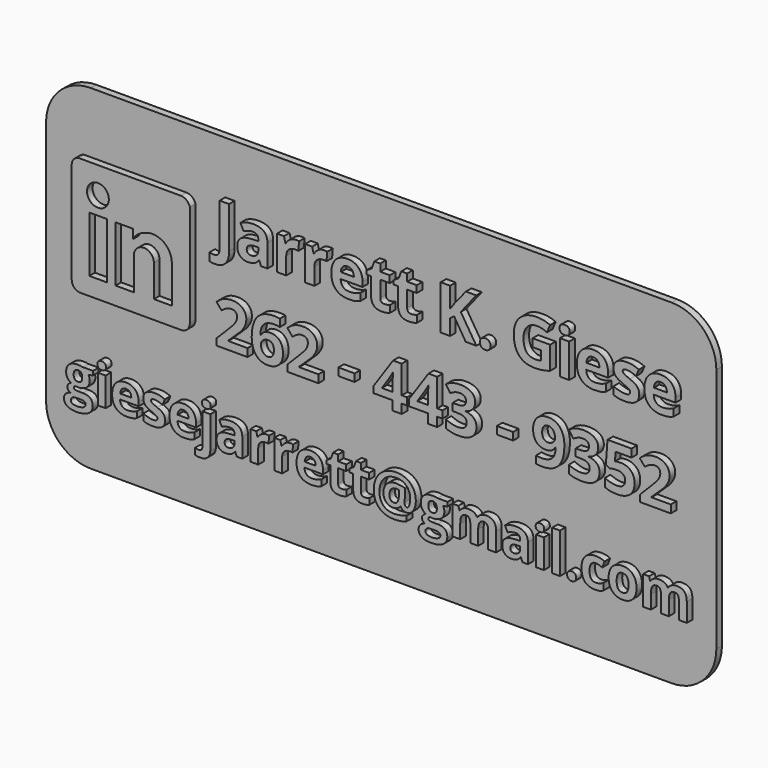
from build123d import *

# Parameters (mm, degrees)
F0_W           = 76.2
F0_H           = 38.1
F0_W_2         = 0.8930238715
F0_H_2         = 3.2741085069
F0_H_3         = 4.5569518229
F0_W_3         = 1.8498784722
F0_H_4         = 0.8609982639
F0_W_4         = 1.0506163194
F0_H_5         = 3.8518923611
F0_R           = 1.2420782833
F0_TEXT_SIZE   = 7.0555555556
F0_TEXT_SIZE_2 = 5.9972222222
F1_DEPTH       = 0.79375
F2_DEPTH       = 0.79375
F3_DEPTH       = 0.79375
F4_DEPTH       = 0.79375
F5_R           = 5.08


# Not quite as in the source:
# - Text() gives the source's letters only with a copy of the font that has no kerning and outlines rounded to 1/6400 em; it was checked with that copy


with BuildPart() as f1:
    # F0 (on Front) → F1 (new body)
    with BuildSketch(Plane.XZ):
        with Locations((-17.37525756, 14.1789878253)):
            Rectangle(F0_W, F0_H)
        with BuildLine():
            Line((-50.6455337371, 5.5282260703), (-49.5032503169, 5.5282260703))
            Line((-49.5032503169, 5.5282260703), (-49.5032503169, 5.0737490738))
            Line((-49.5032503169, 5.0737490738), (-50.0158254038, 4.9425598376))
            add(Edge.make_bspline(
                [(-50.0158254038, 4.9425598376), (-49.8752655079, 4.7223493342), (-49.8752655079, 4.4506002022)],
                knots=[0, 0, 0, 1, 1, 1], degree=2))
            add(Edge.make_bspline(
                [(-49.8752655079, 4.4506002022), (-49.8752655079, 3.9230320599), (-50.243063902, 3.6287933446)],
                knots=[0, 0, 0, 1, 1, 1], degree=2))
            add(Edge.make_bspline(
                [(-50.243063902, 3.6287933446), (-50.6108622961, 3.3345546293), (-51.2630602128, 3.3345546293)],
                knots=[0, 0, 0, 1, 1, 1], degree=2))
            Line((-51.2630602128, 3.3345546293), (-51.42423556, 3.343925289))
            Line((-51.42423556, 3.343925289), (-51.5563618621, 3.3579812786))
            add(Edge.make_bspline(
                [(-51.5563618621, 3.3579812786), (-51.69411056, 3.2530298897), (-51.69411056, 3.1237147856)],
                knots=[0, 0, 0, 1, 1, 1], degree=2))
            add(Edge.make_bspline(
                [(-51.69411056, 3.1237147856), (-51.69411056, 2.9306791953), (-51.2021509246, 2.9306791953)],
                knots=[0, 0, 0, 1, 1, 1], degree=2))
            Line((-51.2021509246, 2.9306791953), (-50.6455337371, 2.9306791953))
            add(Edge.make_bspline(
                [(-50.6455337371, 2.9306791953), (-50.1067208031, 2.9306791953), (-49.8241954124, 2.6992239001)],
                knots=[0, 0, 0, 1, 1, 1], degree=2))
            add(Edge.make_bspline(
                [(-49.8241954124, 2.6992239001), (-49.5416700218, 2.467768605), (-49.5416700218, 2.0198510703)],
                knots=[0, 0, 0, 1, 1, 1], degree=2))
            add(Edge.make_bspline(
                [(-49.5416700218, 2.0198510703), (-49.5416700218, 1.4454296293), (-50.0205107336, 1.1291698637)],
                knots=[0, 0, 0, 1, 1, 1], degree=2))
            add(Edge.make_bspline(
                [(-50.0205107336, 1.1291698637), (-50.4993514454, 0.8129100981), (-51.3951865149, 0.8129100981)],
                knots=[0, 0, 0, 1, 1, 1], degree=2))
            add(Edge.make_bspline(
                [(-51.3951865149, 0.8129100981), (-52.0801817406, 0.8129100981), (-52.4418892058, 1.051861921)],
                knots=[0, 0, 0, 1, 1, 1], degree=2))
            add(Edge.make_bspline(
                [(-52.4418892058, 1.051861921), (-52.8035966711, 1.2908137439), (-52.8035966711, 1.7209270251)],
                knots=[0, 0, 0, 1, 1, 1], degree=2))
            add(Edge.make_bspline(
                [(-52.8035966711, 1.7209270251), (-52.8035966711, 2.0170398724), (-52.6189946746, 2.2161663915)],
                knots=[0, 0, 0, 1, 1, 1], degree=2))
            add(Edge.make_bspline(
                [(-52.6189946746, 2.2161663915), (-52.4343926781, 2.4152929106), (-52.0773705426, 2.500565914)],
                knots=[0, 0, 0, 1, 1, 1], degree=2))
            add(Edge.make_bspline(
                [(-52.0773705426, 2.500565914), (-52.2151192406, 2.5586640043), (-52.3177279645, 2.6917273724)],
                knots=[0, 0, 0, 1, 1, 1], degree=2))
            add(Edge.make_bspline(
                [(-52.3177279645, 2.6917273724), (-52.4203366885, 2.8247907404), (-52.4203366885, 2.974721296)],
                knots=[0, 0, 0, 1, 1, 1], degree=2))
            add(Edge.make_bspline(
                [(-52.4203366885, 2.974721296), (-52.4203366885, 3.1621344904), (-52.3121055687, 3.2862957317)],
                knots=[0, 0, 0, 1, 1, 1], degree=2))
            add(Edge.make_bspline(
                [(-52.3121055687, 3.2862957317), (-52.2038744489, 3.4104569731), (-51.998657001, 3.5313384835)],
                knots=[0, 0, 0, 1, 1, 1], degree=2))
            add(Edge.make_bspline(
                [(-51.998657001, 3.5313384835), (-52.2563501433, 3.6419122682), (-52.4072177649, 3.8878920859)],
                knots=[0, 0, 0, 1, 1, 1], degree=2))
            add(Edge.make_bspline(
                [(-52.4072177649, 3.8878920859), (-52.5580853864, 4.1338719036), (-52.5580853864, 4.4684044557)],
                knots=[0, 0, 0, 1, 1, 1], degree=2))
            add(Edge.make_bspline(
                [(-52.5580853864, 4.4684044557), (-52.5580853864, 5.0034691258), (-52.2094968447, 5.2963022422)],
                knots=[0, 0, 0, 1, 1, 1], degree=2))
            add(Edge.make_bspline(
                [(-52.2094968447, 5.2963022422), (-51.8609083031, 5.5891353585), (-51.2133957163, 5.5891353585)],
                knots=[0, 0, 0, 1, 1, 1], degree=2))
            add(Edge.make_bspline(
                [(-51.2133957163, 5.5891353585), (-51.0756470183, 5.5891353585), (-50.8868282249, 5.5643031102)],
                knots=[0, 0, 0, 1, 1, 1], degree=2))
            add(Edge.make_bspline(
                [(-50.8868282249, 5.5643031102), (-50.6980094315, 5.5394708619), (-50.6455337371, 5.5282260703)],
                knots=[0, 0, 0, 1, 1, 1], degree=2))
        make_face(mode=Mode.SUBTRACT)
        with Locations((-48.5179254472, 3.8911718168)):
            Rectangle(F0_W_2, F0_H_2, mode=Mode.SUBTRACT)
        with BuildLine():
            add(Edge.make_bspline(
                [(-45.0025224524, 2.2522434314), (-45.2686491885, 2.1950824071), (-45.6528462371, 2.1950824071)],
                knots=[0, 0, 0, 1, 1, 1], degree=2))
            add(Edge.make_bspline(
                [(-45.6528462371, 2.1950824071), (-46.4427928517, 2.1950824071), (-46.8878991885, 2.6317551501)],
                knots=[0, 0, 0, 1, 1, 1], degree=2))
            add(Edge.make_bspline(
                [(-46.8878991885, 2.6317551501), (-47.3330055253, 3.0684278932), (-47.3330055253, 3.8677451675)],
                knots=[0, 0, 0, 1, 1, 1], degree=2))
            add(Edge.make_bspline(
                [(-47.3330055253, 3.8677451675), (-47.3330055253, 4.6904890911), (-46.9216335635, 5.1398122248)],
                knots=[0, 0, 0, 1, 1, 1], degree=2))
            add(Edge.make_bspline(
                [(-46.9216335635, 5.1398122248), (-46.5102616017, 5.5891353585), (-45.7840354732, 5.5891353585)],
                knots=[0, 0, 0, 1, 1, 1], degree=2))
            add(Edge.make_bspline(
                [(-45.7840354732, 5.5891353585), (-45.0906066538, 5.5891353585), (-44.7040669402, 5.1941620512)],
                knots=[0, 0, 0, 1, 1, 1], degree=2))
            add(Edge.make_bspline(
                [(-44.7040669402, 5.1941620512), (-44.3175272267, 4.7991887439), (-44.3175272267, 4.1020116606)],
                knots=[0, 0, 0, 1, 1, 1], degree=2))
            Line((-44.3175272267, 4.1020116606), (-44.3175272267, 3.6681501154))
            Line((-44.3175272267, 3.6681501154), (-46.4287368621, 3.6681501154))
            add(Edge.make_bspline(
                [(-46.4287368621, 3.6681501154), (-46.4137438065, 3.2877013307), (-46.2029039628, 3.074050289)],
                knots=[0, 0, 0, 1, 1, 1], degree=2))
            add(Edge.make_bspline(
                [(-46.2029039628, 3.074050289), (-45.992064119, 2.8603992474), (-45.6116153343, 2.8603992474)],
                knots=[0, 0, 0, 1, 1, 1], degree=2))
            add(Edge.make_bspline(
                [(-45.6116153343, 2.8603992474), (-45.3155024871, 2.8603992474), (-45.0521869489, 2.9217770685)],
                knots=[0, 0, 0, 1, 1, 1], degree=2))
            add(Edge.make_bspline(
                [(-45.0521869489, 2.9217770685), (-44.7888714107, 2.9831548897), (-44.5021292232, 3.1180923897)],
                knots=[0, 0, 0, 1, 1, 1], degree=2))
            Line((-44.5021292232, 3.1180923897), (-44.5021292232, 2.4265377022))
            add(Edge.make_bspline(
                [(-44.5021292232, 2.4265377022), (-44.7363957163, 2.3094044557), (-45.0025224524, 2.2522434314)],
                knots=[0, 0, 0, 1, 1, 1], degree=2))
        make_face(mode=Mode.SUBTRACT)
        with BuildLine():
            add(Edge.make_bspline(
                [(-41.3920072614, 3.6451919991), (-41.3067342579, 3.4694921293), (-41.3067342579, 3.2267920425)],
                knots=[0, 0, 0, 1, 1, 1], degree=2))
            add(Edge.make_bspline(
                [(-41.3067342579, 3.2267920425), (-41.3067342579, 2.7226505494), (-41.6567283985, 2.4588664783)],
                knots=[0, 0, 0, 1, 1, 1], degree=2))
            add(Edge.make_bspline(
                [(-41.6567283985, 2.4588664783), (-42.0067225392, 2.1950824071), (-42.7038996225, 2.1950824071)],
                knots=[0, 0, 0, 1, 1, 1], degree=2))
            add(Edge.make_bspline(
                [(-42.7038996225, 2.1950824071), (-43.0609217579, 2.1950824071), (-43.3129925044, 2.2438098376)],
                knots=[0, 0, 0, 1, 1, 1], degree=2))
            add(Edge.make_bspline(
                [(-43.3129925044, 2.2438098376), (-43.565063251, 2.2925372682), (-43.7843366885, 2.3862438654)],
                knots=[0, 0, 0, 1, 1, 1], degree=2))
            Line((-43.7843366885, 2.3862438654), (-43.7843366885, 3.1237147856))
            add(Edge.make_bspline(
                [(-43.7843366885, 3.1237147856), (-43.5360142058, 3.006581539), (-43.2239712371, 2.9273994644)],
                knots=[0, 0, 0, 1, 1, 1], degree=2))
            add(Edge.make_bspline(
                [(-43.2239712371, 2.9273994644), (-42.9119282683, 2.8482173897), (-42.6748505774, 2.8482173897)],
                knots=[0, 0, 0, 1, 1, 1], degree=2))
            add(Edge.make_bspline(
                [(-42.6748505774, 2.8482173897), (-42.1885133378, 2.8482173897), (-42.1885133378, 3.1293371814)],
                knots=[0, 0, 0, 1, 1, 1], degree=2))
            add(Edge.make_bspline(
                [(-42.1885133378, 3.1293371814), (-42.1885133378, 3.2352256363), (-42.2531708899, 3.3012887873)],
                knots=[0, 0, 0, 1, 1, 1], degree=2))
            add(Edge.make_bspline(
                [(-42.2531708899, 3.3012887873), (-42.3178284419, 3.3673519383), (-42.4757240583, 3.4507508099)],
                knots=[0, 0, 0, 1, 1, 1], degree=2))
            add(Edge.make_bspline(
                [(-42.4757240583, 3.4507508099), (-42.6336196746, 3.5341496814), (-42.8969352128, 3.6447234661)],
                knots=[0, 0, 0, 1, 1, 1], degree=2))
            add(Edge.make_bspline(
                [(-42.8969352128, 3.6447234661), (-43.2745727996, 3.8030876154), (-43.4521468013, 3.9380251154)],
                knots=[0, 0, 0, 1, 1, 1], degree=2))
            add(Edge.make_bspline(
                [(-43.4521468013, 3.9380251154), (-43.6297208031, 4.0729626154), (-43.7098399437, 4.2472568863)],
                knots=[0, 0, 0, 1, 1, 1], degree=2))
            add(Edge.make_bspline(
                [(-43.7098399437, 4.2472568863), (-43.7899590843, 4.4215511571), (-43.7899590843, 4.6754960356)],
                knots=[0, 0, 0, 1, 1, 1], degree=2))
            add(Edge.make_bspline(
                [(-43.7899590843, 4.6754960356), (-43.7899590843, 5.1121687786), (-43.4521468013, 5.3506520685)],
                knots=[0, 0, 0, 1, 1, 1], degree=2))
            add(Edge.make_bspline(
                [(-43.4521468013, 5.3506520685), (-43.1143345183, 5.5891353585), (-42.4930597788, 5.5891353585)],
                knots=[0, 0, 0, 1, 1, 1], degree=2))
            add(Edge.make_bspline(
                [(-42.4930597788, 5.5891353585), (-41.9017711503, 5.5891353585), (-41.3423427649, 5.3314422161)],
                knots=[0, 0, 0, 1, 1, 1], degree=2))
            Line((-41.3423427649, 5.3314422161), (-41.6112806989, 4.6876778932))
            add(Edge.make_bspline(
                [(-41.6112806989, 4.6876778932), (-41.8577290496, 4.7926292821), (-42.0713800913, 4.8600980321)],
                knots=[0, 0, 0, 1, 1, 1], degree=2))
            add(Edge.make_bspline(
                [(-42.0713800913, 4.8600980321), (-42.2850311329, 4.9275667821), (-42.5080528343, 4.9275667821)],
                knots=[0, 0, 0, 1, 1, 1], degree=2))
            add(Edge.make_bspline(
                [(-42.5080528343, 4.9275667821), (-42.9034946746, 4.9275667821), (-42.9034946746, 4.7139157404)],
                knots=[0, 0, 0, 1, 1, 1], degree=2))
            add(Edge.make_bspline(
                [(-42.9034946746, 4.7139157404), (-42.9034946746, 4.593971296), (-42.7760537024, 4.5058870946)],
                knots=[0, 0, 0, 1, 1, 1], degree=2))
            add(Edge.make_bspline(
                [(-42.7760537024, 4.5058870946), (-42.6486127301, 4.4178028932), (-42.2175623829, 4.2453827543)],
                knots=[0, 0, 0, 1, 1, 1], degree=2))
            add(Edge.make_bspline(
                [(-42.2175623829, 4.2453827543), (-41.8343024003, 4.0898298029), (-41.6557913326, 3.9553608359)],
                knots=[0, 0, 0, 1, 1, 1], degree=2))
            add(Edge.make_bspline(
                [(-41.6557913326, 3.9553608359), (-41.4772802649, 3.8208918689), (-41.3920072614, 3.6451919991)],
                knots=[0, 0, 0, 1, 1, 1], degree=2))
        make_face(mode=Mode.SUBTRACT)
        with BuildLine():
            add(Edge.make_bspline(
                [(-36.4761591711, 1.0959040217), (-36.7778944142, 0.8129100981), (-37.3307633378, 0.8129100981)],
                knots=[0, 0, 0, 1, 1, 1], degree=2))
            add(Edge.make_bspline(
                [(-37.3307633378, 0.8129100981), (-37.6737294836, 0.8129100981), (-37.9192407683, 0.8869383099)],
                knots=[0, 0, 0, 1, 1, 1], degree=2))
            Line((-37.9192407683, 0.8869383099), (-37.9192407683, 1.589737789))
            add(Edge.make_bspline(
                [(-37.9192407683, 1.589737789), (-37.7149603864, 1.5335138307), (-37.5003722788, 1.5335138307)],
                knots=[0, 0, 0, 1, 1, 1], degree=2))
            add(Edge.make_bspline(
                [(-37.5003722788, 1.5335138307), (-37.2754764454, 1.5335138307), (-37.1714621225, 1.659549204)],
                knots=[0, 0, 0, 1, 1, 1], degree=2))
            add(Edge.make_bspline(
                [(-37.1714621225, 1.659549204), (-37.0674477996, 1.7855845772), (-37.0674477996, 2.0310958619)],
                knots=[0, 0, 0, 1, 1, 1], degree=2))
            Line((-37.0674477996, 2.0310958619), (-37.0674477996, 5.5282260703))
            Line((-37.0674477996, 5.5282260703), (-36.1744239281, 5.5282260703))
            Line((-36.1744239281, 5.5282260703), (-36.1744239281, 1.8999066258))
            add(Edge.make_bspline(
                [(-36.1744239281, 1.8999066258), (-36.1744239281, 1.3788979453), (-36.4761591711, 1.0959040217)],
                knots=[0, 0, 0, 1, 1, 1], degree=2))
        make_face(mode=Mode.SUBTRACT)
        with BuildLine():
            add(Edge.make_bspline(
                [(-38.4786691538, 2.2522434314), (-38.7447958899, 2.1950824071), (-39.1289929385, 2.1950824071)],
                knots=[0, 0, 0, 1, 1, 1], degree=2))
            add(Edge.make_bspline(
                [(-39.1289929385, 2.1950824071), (-39.9189395531, 2.1950824071), (-40.3640458899, 2.6317551501)],
                knots=[0, 0, 0, 1, 1, 1], degree=2))
            add(Edge.make_bspline(
                [(-40.3640458899, 2.6317551501), (-40.8091522267, 3.0684278932), (-40.8091522267, 3.8677451675)],
                knots=[0, 0, 0, 1, 1, 1], degree=2))
            add(Edge.make_bspline(
                [(-40.8091522267, 3.8677451675), (-40.8091522267, 4.6904890911), (-40.3977802649, 5.1398122248)],
                knots=[0, 0, 0, 1, 1, 1], degree=2))
            add(Edge.make_bspline(
                [(-40.3977802649, 5.1398122248), (-39.9864083031, 5.5891353585), (-39.2601821746, 5.5891353585)],
                knots=[0, 0, 0, 1, 1, 1], degree=2))
            add(Edge.make_bspline(
                [(-39.2601821746, 5.5891353585), (-38.5667533551, 5.5891353585), (-38.1802136416, 5.1941620512)],
                knots=[0, 0, 0, 1, 1, 1], degree=2))
            add(Edge.make_bspline(
                [(-38.1802136416, 5.1941620512), (-37.7936739281, 4.7991887439), (-37.7936739281, 4.1020116606)],
                knots=[0, 0, 0, 1, 1, 1], degree=2))
            Line((-37.7936739281, 4.1020116606), (-37.7936739281, 3.6681501154))
            Line((-37.7936739281, 3.6681501154), (-39.9048835635, 3.6681501154))
            add(Edge.make_bspline(
                [(-39.9048835635, 3.6681501154), (-39.8898905079, 3.2877013307), (-39.6790506642, 3.074050289)],
                knots=[0, 0, 0, 1, 1, 1], degree=2))
            add(Edge.make_bspline(
                [(-39.6790506642, 3.074050289), (-39.4682108204, 2.8603992474), (-39.0877620357, 2.8603992474)],
                knots=[0, 0, 0, 1, 1, 1], degree=2))
            add(Edge.make_bspline(
                [(-39.0877620357, 2.8603992474), (-38.7916491885, 2.8603992474), (-38.5283336503, 2.9217770685)],
                knots=[0, 0, 0, 1, 1, 1], degree=2))
            add(Edge.make_bspline(
                [(-38.5283336503, 2.9217770685), (-38.2650181121, 2.9831548897), (-37.9782759246, 3.1180923897)],
                knots=[0, 0, 0, 1, 1, 1], degree=2))
            Line((-37.9782759246, 3.1180923897), (-37.9782759246, 2.4265377022))
            add(Edge.make_bspline(
                [(-37.9782759246, 2.4265377022), (-38.2125424176, 2.3094044557), (-38.4786691538, 2.2522434314)],
                knots=[0, 0, 0, 1, 1, 1], degree=2))
        make_face(mode=Mode.SUBTRACT)
        with BuildLine():
            Line((-32.5348596919, 2.2541175633), (-33.1580085635, 2.2541175633))
            Line((-33.1580085635, 2.2541175633), (-33.3313657683, 2.6992239001))
            Line((-33.3313657683, 2.6992239001), (-33.3547924176, 2.6992239001))
            add(Edge.make_bspline(
                [(-33.3547924176, 2.6992239001), (-33.579688251, 2.4152929106), (-33.8186400739, 2.3051876588)],
                knots=[0, 0, 0, 1, 1, 1], degree=2))
            add(Edge.make_bspline(
                [(-33.8186400739, 2.3051876588), (-34.0575918968, 2.1950824071), (-34.4408518794, 2.1950824071)],
                knots=[0, 0, 0, 1, 1, 1], degree=2))
            add(Edge.make_bspline(
                [(-34.4408518794, 2.1950824071), (-34.9121960635, 2.1950824071), (-35.1830081294, 2.4649574071)],
                knots=[0, 0, 0, 1, 1, 1], degree=2))
            add(Edge.make_bspline(
                [(-35.1830081294, 2.4649574071), (-35.4538201954, 2.7348324071), (-35.4538201954, 3.2324144383)],
                knots=[0, 0, 0, 1, 1, 1], degree=2))
            add(Edge.make_bspline(
                [(-35.4538201954, 3.2324144383), (-35.4538201954, 3.7534231189), (-35.0893015322, 4.0008085356)],
                knots=[0, 0, 0, 1, 1, 1], degree=2))
            add(Edge.make_bspline(
                [(-35.0893015322, 4.0008085356), (-34.724782869, 4.2481939522), (-33.9901231468, 4.2744317994)],
                knots=[0, 0, 0, 1, 1, 1], degree=2))
            Line((-33.9901231468, 4.2744317994), (-33.4213241017, 4.2922360529))
            Line((-33.4213241017, 4.2922360529), (-33.4213241017, 4.4356071467))
            add(Edge.make_bspline(
                [(-33.4213241017, 4.4356071467), (-33.4213241017, 4.9331891779), (-33.9310879906, 4.9331891779)],
                knots=[0, 0, 0, 1, 1, 1], degree=2))
            add(Edge.make_bspline(
                [(-33.9310879906, 4.9331891779), (-34.3237186329, 4.9331891779), (-34.8540979732, 4.6961114869)],
                knots=[0, 0, 0, 1, 1, 1], degree=2))
            Line((-34.8540979732, 4.6961114869), (-35.1492737544, 5.2995819731))
            add(Edge.make_bspline(
                [(-35.1492737544, 5.2995819731), (-34.5842229732, 5.5956948203), (-33.8964165496, 5.5956948203)],
                knots=[0, 0, 0, 1, 1, 1], degree=2))
            add(Edge.make_bspline(
                [(-33.8964165496, 5.5956948203), (-33.2376591711, 5.5956948203), (-32.8862594315, 5.3084840998)],
                knots=[0, 0, 0, 1, 1, 1], degree=2))
            add(Edge.make_bspline(
                [(-32.8862594315, 5.3084840998), (-32.5348596919, 5.0212733793), (-32.5348596919, 4.4356071467)],
                knots=[0, 0, 0, 1, 1, 1], degree=2))
            Line((-32.5348596919, 4.4356071467), (-32.5348596919, 2.2541175633))
        make_face(mode=Mode.SUBTRACT)
        with BuildLine():
            add(Edge.make_bspline(
                [(-30.3510274437, 5.4209320165), (-30.0919287024, 5.5891353585), (-29.7873822614, 5.5891353585)],
                knots=[0, 0, 0, 1, 1, 1], degree=2))
            add(Edge.make_bspline(
                [(-29.7873822614, 5.5891353585), (-29.6055914628, 5.5891353585), (-29.4856470183, 5.5628975113)],
                knots=[0, 0, 0, 1, 1, 1], degree=2))
            Line((-29.4856470183, 5.5628975113), (-29.5531157683, 4.7260975981))
            add(Edge.make_bspline(
                [(-29.5531157683, 4.7260975981), (-29.6618154211, 4.7551466432), (-29.8164313065, 4.7551466432)],
                knots=[0, 0, 0, 1, 1, 1], degree=2))
            add(Edge.make_bspline(
                [(-29.8164313065, 4.7551466432), (-30.2437333899, 4.7551466432), (-30.4826852128, 4.5354046727)],
                knots=[0, 0, 0, 1, 1, 1], degree=2))
            add(Edge.make_bspline(
                [(-30.4826852128, 4.5354046727), (-30.7216370357, 4.3156627022), (-30.7216370357, 3.9202208619)],
                knots=[0, 0, 0, 1, 1, 1], degree=2))
            Line((-30.7216370357, 3.9202208619), (-30.7216370357, 2.2541175633))
            Line((-30.7216370357, 2.2541175633), (-31.6146609072, 2.2541175633))
            Line((-31.6146609072, 2.2541175633), (-31.6146609072, 5.5282260703))
            Line((-31.6146609072, 5.5282260703), (-30.9380992753, 5.5282260703))
            Line((-30.9380992753, 5.5282260703), (-30.8059729732, 4.9772312786))
            Line((-30.8059729732, 4.9772312786), (-30.7628679385, 4.9772312786))
            add(Edge.make_bspline(
                [(-30.7628679385, 4.9772312786), (-30.610126185, 5.2527286744), (-30.3510274437, 5.4209320165)],
                knots=[0, 0, 0, 1, 1, 1], degree=2))
        make_face(mode=Mode.SUBTRACT)
        with BuildLine():
            add(Edge.make_bspline(
                [(-27.6279137284, 5.4209320165), (-27.3688149871, 5.5891353585), (-27.0642685461, 5.5891353585)],
                knots=[0, 0, 0, 1, 1, 1], degree=2))
            add(Edge.make_bspline(
                [(-27.0642685461, 5.5891353585), (-26.8824777475, 5.5891353585), (-26.7625333031, 5.5628975113)],
                knots=[0, 0, 0, 1, 1, 1], degree=2))
            Line((-26.7625333031, 5.5628975113), (-26.8300020531, 4.7260975981))
            add(Edge.make_bspline(
                [(-26.8300020531, 4.7260975981), (-26.9387017058, 4.7551466432), (-27.0933175913, 4.7551466432)],
                knots=[0, 0, 0, 1, 1, 1], degree=2))
            add(Edge.make_bspline(
                [(-27.0933175913, 4.7551466432), (-27.5206196746, 4.7551466432), (-27.7595714975, 4.5354046727)],
                knots=[0, 0, 0, 1, 1, 1], degree=2))
            add(Edge.make_bspline(
                [(-27.7595714975, 4.5354046727), (-27.9985233204, 4.3156627022), (-27.9985233204, 3.9202208619)],
                knots=[0, 0, 0, 1, 1, 1], degree=2))
            Line((-27.9985233204, 3.9202208619), (-27.9985233204, 2.2541175633))
            Line((-27.9985233204, 2.2541175633), (-28.8915471919, 2.2541175633))
            Line((-28.8915471919, 2.2541175633), (-28.8915471919, 5.5282260703))
            Line((-28.8915471919, 5.5282260703), (-28.21498556, 5.5282260703))
            Line((-28.21498556, 5.5282260703), (-28.0828592579, 4.9772312786))
            Line((-28.0828592579, 4.9772312786), (-28.0397542232, 4.9772312786))
            add(Edge.make_bspline(
                [(-28.0397542232, 4.9772312786), (-27.8870124697, 5.2527286744), (-27.6279137284, 5.4209320165)],
                knots=[0, 0, 0, 1, 1, 1], degree=2))
        make_face(mode=Mode.SUBTRACT)
        with BuildLine():
            add(Edge.make_bspline(
                [(-24.0366083899, 2.2522434314), (-24.302735126, 2.1950824071), (-24.6869321746, 2.1950824071)],
                knots=[0, 0, 0, 1, 1, 1], degree=2))
            add(Edge.make_bspline(
                [(-24.6869321746, 2.1950824071), (-25.4768787892, 2.1950824071), (-25.921985126, 2.6317551501)],
                knots=[0, 0, 0, 1, 1, 1], degree=2))
            add(Edge.make_bspline(
                [(-25.921985126, 2.6317551501), (-26.3670914628, 3.0684278932), (-26.3670914628, 3.8677451675)],
                knots=[0, 0, 0, 1, 1, 1], degree=2))
            add(Edge.make_bspline(
                [(-26.3670914628, 3.8677451675), (-26.3670914628, 4.6904890911), (-25.955719501, 5.1398122248)],
                knots=[0, 0, 0, 1, 1, 1], degree=2))
            add(Edge.make_bspline(
                [(-25.955719501, 5.1398122248), (-25.5443475392, 5.5891353585), (-24.8181214107, 5.5891353585)],
                knots=[0, 0, 0, 1, 1, 1], degree=2))
            add(Edge.make_bspline(
                [(-24.8181214107, 5.5891353585), (-24.1246925913, 5.5891353585), (-23.7381528777, 5.1941620512)],
                knots=[0, 0, 0, 1, 1, 1], degree=2))
            add(Edge.make_bspline(
                [(-23.7381528777, 5.1941620512), (-23.3516131642, 4.7991887439), (-23.3516131642, 4.1020116606)],
                knots=[0, 0, 0, 1, 1, 1], degree=2))
            Line((-23.3516131642, 4.1020116606), (-23.3516131642, 3.6681501154))
            Line((-23.3516131642, 3.6681501154), (-25.4628227996, 3.6681501154))
            add(Edge.make_bspline(
                [(-25.4628227996, 3.6681501154), (-25.447829744, 3.2877013307), (-25.2369899003, 3.074050289)],
                knots=[0, 0, 0, 1, 1, 1], degree=2))
            add(Edge.make_bspline(
                [(-25.2369899003, 3.074050289), (-25.0261500565, 2.8603992474), (-24.6457012718, 2.8603992474)],
                knots=[0, 0, 0, 1, 1, 1], degree=2))
            add(Edge.make_bspline(
                [(-24.6457012718, 2.8603992474), (-24.3495884246, 2.8603992474), (-24.0862728864, 2.9217770685)],
                knots=[0, 0, 0, 1, 1, 1], degree=2))
            add(Edge.make_bspline(
                [(-24.0862728864, 2.9217770685), (-23.8229573482, 2.9831548897), (-23.5362151607, 3.1180923897)],
                knots=[0, 0, 0, 1, 1, 1], degree=2))
            Line((-23.5362151607, 3.1180923897), (-23.5362151607, 2.4265377022))
            add(Edge.make_bspline(
                [(-23.5362151607, 2.4265377022), (-23.7704816538, 2.3094044557), (-24.0366083899, 2.2522434314)],
                knots=[0, 0, 0, 1, 1, 1], degree=2))
        make_face(mode=Mode.SUBTRACT)
        with BuildLine():
            add(Edge.make_bspline(
                [(-21.5290198482, 2.9981479453), (-21.4221943274, 2.907252546), (-21.2460259246, 2.907252546)],
                knots=[0, 0, 0, 1, 1, 1], degree=2))
            add(Edge.make_bspline(
                [(-21.2460259246, 2.907252546), (-21.0117594315, 2.907252546), (-20.6837863413, 3.0093927369)],
                knots=[0, 0, 0, 1, 1, 1], degree=2))
            Line((-20.6837863413, 3.0093927369), (-20.6837863413, 2.3450129626))
            add(Edge.make_bspline(
                [(-20.6837863413, 2.3450129626), (-21.0173818274, 2.1950824071), (-21.5037190669, 2.1950824071)],
                knots=[0, 0, 0, 1, 1, 1], degree=2))
            add(Edge.make_bspline(
                [(-21.5037190669, 2.1950824071), (-22.0397208031, 2.1950824071), (-22.2842950218, 2.466363006)],
                knots=[0, 0, 0, 1, 1, 1], degree=2))
            add(Edge.make_bspline(
                [(-22.2842950218, 2.466363006), (-22.5288692406, 2.737643605), (-22.5288692406, 3.2792677369)],
                knots=[0, 0, 0, 1, 1, 1], degree=2))
            Line((-22.5288692406, 3.2792677369), (-22.5288692406, 4.8572868342))
            Line((-22.5288692406, 4.8572868342), (-22.9561713239, 4.8572868342))
            Line((-22.9561713239, 4.8572868342), (-22.9561713239, 5.234924421))
            Line((-22.9561713239, 5.234924421), (-22.4642116885, 5.5338484661))
            Line((-22.4642116885, 5.5338484661), (-22.2065185461, 6.2254031536))
            Line((-22.2065185461, 6.2254031536), (-21.635845369, 6.2254031536))
            Line((-21.635845369, 6.2254031536), (-21.635845369, 5.5282260703))
            Line((-21.635845369, 5.5282260703), (-20.7193948482, 5.5282260703))
            Line((-20.7193948482, 5.5282260703), (-20.7193948482, 4.8572868342))
            Line((-20.7193948482, 4.8572868342), (-21.635845369, 4.8572868342))
            Line((-21.635845369, 4.8572868342), (-21.635845369, 3.2792677369))
            add(Edge.make_bspline(
                [(-21.635845369, 3.2792677369), (-21.635845369, 3.0890433446), (-21.5290198482, 2.9981479453)],
                knots=[0, 0, 0, 1, 1, 1], degree=2))
        make_face(mode=Mode.SUBTRACT)
        with BuildLine():
            add(Edge.make_bspline(
                [(-18.9258505774, 2.9981479453), (-18.8190250565, 2.907252546), (-18.6428566538, 2.907252546)],
                knots=[0, 0, 0, 1, 1, 1], degree=2))
            add(Edge.make_bspline(
                [(-18.6428566538, 2.907252546), (-18.4085901607, 2.907252546), (-18.0806170704, 3.0093927369)],
                knots=[0, 0, 0, 1, 1, 1], degree=2))
            Line((-18.0806170704, 3.0093927369), (-18.0806170704, 2.3450129626))
            add(Edge.make_bspline(
                [(-18.0806170704, 2.3450129626), (-18.4142125565, 2.1950824071), (-18.9005497961, 2.1950824071)],
                knots=[0, 0, 0, 1, 1, 1], degree=2))
            add(Edge.make_bspline(
                [(-18.9005497961, 2.1950824071), (-19.4365515322, 2.1950824071), (-19.681125751, 2.466363006)],
                knots=[0, 0, 0, 1, 1, 1], degree=2))
            add(Edge.make_bspline(
                [(-19.681125751, 2.466363006), (-19.9256999697, 2.737643605), (-19.9256999697, 3.2792677369)],
                knots=[0, 0, 0, 1, 1, 1], degree=2))
            Line((-19.9256999697, 3.2792677369), (-19.9256999697, 4.8572868342))
            Line((-19.9256999697, 4.8572868342), (-20.3530020531, 4.8572868342))
            Line((-20.3530020531, 4.8572868342), (-20.3530020531, 5.234924421))
            Line((-20.3530020531, 5.234924421), (-19.8610424176, 5.5338484661))
            Line((-19.8610424176, 5.5338484661), (-19.6033492753, 6.2254031536))
            Line((-19.6033492753, 6.2254031536), (-19.0326760982, 6.2254031536))
            Line((-19.0326760982, 6.2254031536), (-19.0326760982, 5.5282260703))
            Line((-19.0326760982, 5.5282260703), (-18.1162255774, 5.5282260703))
            Line((-18.1162255774, 5.5282260703), (-18.1162255774, 4.8572868342))
            Line((-18.1162255774, 4.8572868342), (-19.0326760982, 4.8572868342))
            Line((-19.0326760982, 4.8572868342), (-19.0326760982, 3.2792677369))
            add(Edge.make_bspline(
                [(-19.0326760982, 3.2792677369), (-19.0326760982, 3.0890433446), (-18.9258505774, 2.9981479453)],
                knots=[0, 0, 0, 1, 1, 1], degree=2))
        make_face(mode=Mode.SUBTRACT)
        with BuildLine():
            add(Edge.make_bspline(
                [(-48.5165198482, 5.9349127022), (-49.0028570878, 5.9349127022), (-49.0028570878, 6.3743966432)],
                knots=[0, 0, 0, 1, 1, 1], degree=2))
            add(Edge.make_bspline(
                [(-49.0028570878, 6.3743966432), (-49.0028570878, 6.8110693863), (-48.5165198482, 6.8110693863)],
                knots=[0, 0, 0, 1, 1, 1], degree=2))
            add(Edge.make_bspline(
                [(-48.5165198482, 6.8110693863), (-48.0301826086, 6.8110693863), (-48.0301826086, 6.3743966432)],
                knots=[0, 0, 0, 1, 1, 1], degree=2))
            add(Edge.make_bspline(
                [(-48.0301826086, 6.3743966432), (-48.0301826086, 6.1663679974), (-48.151532652, 6.0506403498)],
                knots=[0, 0, 0, 1, 1, 1], degree=2))
            add(Edge.make_bspline(
                [(-48.151532652, 6.0506403498), (-48.2728826954, 5.9349127022), (-48.5165198482, 5.9349127022)],
                knots=[0, 0, 0, 1, 1, 1], degree=2))
        make_face(mode=Mode.SUBTRACT)
        with BuildLine():
            add(Edge.make_bspline(
                [(-36.6195302649, 5.9349127022), (-37.1058675044, 5.9349127022), (-37.1058675044, 6.3743966432)],
                knots=[0, 0, 0, 1, 1, 1], degree=2))
            add(Edge.make_bspline(
                [(-37.1058675044, 6.3743966432), (-37.1058675044, 6.8110693863), (-36.6195302649, 6.8110693863)],
                knots=[0, 0, 0, 1, 1, 1], degree=2))
            add(Edge.make_bspline(
                [(-36.6195302649, 6.8110693863), (-36.1331930253, 6.8110693863), (-36.1331930253, 6.3743966432)],
                knots=[0, 0, 0, 1, 1, 1], degree=2))
            add(Edge.make_bspline(
                [(-36.1331930253, 6.3743966432), (-36.1331930253, 6.1663679974), (-36.2545430687, 6.0506403498)],
                knots=[0, 0, 0, 1, 1, 1], degree=2))
            add(Edge.make_bspline(
                [(-36.2545430687, 6.0506403498), (-36.3758931121, 5.9349127022), (-36.6195302649, 5.9349127022)],
                knots=[0, 0, 0, 1, 1, 1], degree=2))
        make_face(mode=Mode.SUBTRACT)
        with BuildLine():
            add(Edge.make_bspline(
                [(-13.0823071746, 5.5778905668), (-12.8068097788, 5.0915533272), (-12.8068097788, 4.4562225981)],
                knots=[0, 0, 0, 1, 1, 1], degree=2))
            add(Edge.make_bspline(
                [(-12.8068097788, 4.4562225981), (-12.8068097788, 4.0345429106), (-12.9417472788, 3.6845487699)],
                knots=[0, 0, 0, 1, 1, 1], degree=2))
            add(Edge.make_bspline(
                [(-12.9417472788, 3.6845487699), (-13.0766847788, 3.3345546293), (-13.3226645965, 3.1354281102)],
                knots=[0, 0, 0, 1, 1, 1], degree=2))
            add(Edge.make_bspline(
                [(-13.3226645965, 3.1354281102), (-13.5686444142, 2.9363015911), (-13.8928692406, 2.9363015911)],
                knots=[0, 0, 0, 1, 1, 1], degree=2))
            add(Edge.make_bspline(
                [(-13.8928692406, 2.9363015911), (-14.1102685461, 2.9363015911), (-14.2770662892, 3.040315914)],
                knots=[0, 0, 0, 1, 1, 1], degree=2))
            add(Edge.make_bspline(
                [(-14.2770662892, 3.040315914), (-14.4438640322, 3.1443302369), (-14.5169551781, 3.3139391779)],
                knots=[0, 0, 0, 1, 1, 1], degree=2))
            Line((-14.5169551781, 3.3139391779), (-14.5638084767, 3.3139391779))
            add(Edge.make_bspline(
                [(-14.5638084767, 3.3139391779), (-14.8805367753, 2.9363015911), (-15.3687481468, 2.9363015911)],
                knots=[0, 0, 0, 1, 1, 1], degree=2))
            add(Edge.make_bspline(
                [(-15.3687481468, 2.9363015911), (-15.8878826954, 2.9363015911), (-16.1863382076, 3.2483445599)],
                knots=[0, 0, 0, 1, 1, 1], degree=2))
            add(Edge.make_bspline(
                [(-16.1863382076, 3.2483445599), (-16.4847937197, 3.5603875286), (-16.4847937197, 4.1020116606)],
                knots=[0, 0, 0, 1, 1, 1], degree=2))
            add(Edge.make_bspline(
                [(-16.4847937197, 4.1020116606), (-16.4847937197, 4.7195381363), (-16.0926316103, 5.097644256)],
                knots=[0, 0, 0, 1, 1, 1], degree=2))
            add(Edge.make_bspline(
                [(-16.0926316103, 5.097644256), (-15.700469501, 5.4757503758), (-15.0679499697, 5.4757503758)],
                knots=[0, 0, 0, 1, 1, 1], degree=2))
            add(Edge.make_bspline(
                [(-15.0679499697, 5.4757503758), (-14.8158792232, 5.4757503758), (-14.5127383812, 5.4270229453)],
                knots=[0, 0, 0, 1, 1, 1], degree=2))
            add(Edge.make_bspline(
                [(-14.5127383812, 5.4270229453), (-14.2095975392, 5.3782955147), (-14.013750751, 5.3117638307)],
                knots=[0, 0, 0, 1, 1, 1], degree=2))
            Line((-14.013750751, 5.3117638307), (-14.080282435, 3.8789899592))
            add(Edge.make_bspline(
                [(-14.080282435, 3.8789899592), (-14.080282435, 3.4723033272), (-13.8581977996, 3.4723033272)],
                knots=[0, 0, 0, 1, 1, 1], degree=2))
            add(Edge.make_bspline(
                [(-13.8581977996, 3.4723033272), (-13.6707846051, 3.4723033272), (-13.5592737544, 3.7459265911)],
                knots=[0, 0, 0, 1, 1, 1], degree=2))
            add(Edge.make_bspline(
                [(-13.5592737544, 3.7459265911), (-13.4477629038, 4.019549855), (-13.4477629038, 4.4618449939)],
                knots=[0, 0, 0, 1, 1, 1], degree=2))
            add(Edge.make_bspline(
                [(-13.4477629038, 4.4618449939), (-13.4477629038, 4.9331891779), (-13.6440782249, 5.2948966432)],
                knots=[0, 0, 0, 1, 1, 1], degree=2))
            add(Edge.make_bspline(
                [(-13.6440782249, 5.2948966432), (-13.8403935461, 5.6566041085), (-14.1964786156, 5.8472970338)],
                knots=[0, 0, 0, 1, 1, 1], degree=2))
            add(Edge.make_bspline(
                [(-14.1964786156, 5.8472970338), (-14.552563685, 6.0379899592), (-15.0089148135, 6.0379899592)],
                knots=[0, 0, 0, 1, 1, 1], degree=2))
            add(Edge.make_bspline(
                [(-15.0089148135, 6.0379899592), (-15.6002034419, 6.0379899592), (-16.036876185, 5.7948213394)],
                knots=[0, 0, 0, 1, 1, 1], degree=2))
            add(Edge.make_bspline(
                [(-16.036876185, 5.7948213394), (-16.4735489281, 5.5516527196), (-16.7059412892, 5.0934274592)],
                knots=[0, 0, 0, 1, 1, 1], degree=2))
            add(Edge.make_bspline(
                [(-16.7059412892, 5.0934274592), (-16.9383336503, 4.6352021988), (-16.9383336503, 4.0345429106)],
                knots=[0, 0, 0, 1, 1, 1], degree=2))
            add(Edge.make_bspline(
                [(-16.9383336503, 4.0345429106), (-16.9383336503, 3.2267920425), (-16.5068147701, 2.7948046293)],
                knots=[0, 0, 0, 1, 1, 1], degree=2))
            add(Edge.make_bspline(
                [(-16.5068147701, 2.7948046293), (-16.0752958899, 2.3628172161), (-15.2553631642, 2.3628172161)],
                knots=[0, 0, 0, 1, 1, 1], degree=2))
            add(Edge.make_bspline(
                [(-15.2553631642, 2.3628172161), (-14.9442572614, 2.3628172161), (-14.5727106034, 2.4316915651)],
                knots=[0, 0, 0, 1, 1, 1], degree=2))
            add(Edge.make_bspline(
                [(-14.5727106034, 2.4316915651), (-14.2011639454, 2.500565914), (-13.8403935461, 2.6317551501)],
                knots=[0, 0, 0, 1, 1, 1], degree=2))
            Line((-13.8403935461, 2.6317551501), (-13.8403935461, 2.0695155668))
            add(Edge.make_bspline(
                [(-13.8403935461, 2.0695155668), (-14.4672906815, 1.8033888307), (-15.2319365149, 1.8033888307)],
                knots=[0, 0, 0, 1, 1, 1], degree=2))
            add(Edge.make_bspline(
                [(-15.2319365149, 1.8033888307), (-16.3442338239, 1.8033888307), (-16.9664456294, 2.3890550633)],
                knots=[0, 0, 0, 1, 1, 1], degree=2))
            add(Edge.make_bspline(
                [(-16.9664456294, 2.3890550633), (-17.588657435, 2.974721296), (-17.588657435, 4.0167386571)],
                knots=[0, 0, 0, 1, 1, 1], degree=2))
            add(Edge.make_bspline(
                [(-17.588657435, 4.0167386571), (-17.588657435, 4.7401535876), (-17.2709920704, 5.3305051501)],
                knots=[0, 0, 0, 1, 1, 1], degree=2))
            add(Edge.make_bspline(
                [(-17.2709920704, 5.3305051501), (-16.9533267058, 5.9208567126), (-16.3662548742, 6.2558577977)],
                knots=[0, 0, 0, 1, 1, 1], degree=2))
            add(Edge.make_bspline(
                [(-16.3662548742, 6.2558577977), (-15.7791830426, 6.5908588828), (-15.0145372093, 6.5908588828)],
                knots=[0, 0, 0, 1, 1, 1], degree=2))
            add(Edge.make_bspline(
                [(-15.0145372093, 6.5908588828), (-14.3707728864, 6.5908588828), (-13.8642887284, 6.3275433446)],
                knots=[0, 0, 0, 1, 1, 1], degree=2))
            add(Edge.make_bspline(
                [(-13.8642887284, 6.3275433446), (-13.3578045704, 6.0642278064), (-13.0823071746, 5.5778905668)],
                knots=[0, 0, 0, 1, 1, 1], degree=2))
        make_face(mode=Mode.SUBTRACT)
        with BuildLine():
            Line((-10.3320185461, 5.5282260703), (-9.189735126, 5.5282260703))
            Line((-9.189735126, 5.5282260703), (-9.189735126, 5.0737490738))
            Line((-9.189735126, 5.0737490738), (-9.7023102128, 4.9425598376))
            add(Edge.make_bspline(
                [(-9.7023102128, 4.9425598376), (-9.5617503169, 4.7223493342), (-9.5617503169, 4.4506002022)],
                knots=[0, 0, 0, 1, 1, 1], degree=2))
            add(Edge.make_bspline(
                [(-9.5617503169, 4.4506002022), (-9.5617503169, 3.9230320599), (-9.929548711, 3.6287933446)],
                knots=[0, 0, 0, 1, 1, 1], degree=2))
            add(Edge.make_bspline(
                [(-9.929548711, 3.6287933446), (-10.2973471051, 3.3345546293), (-10.9495450218, 3.3345546293)],
                knots=[0, 0, 0, 1, 1, 1], degree=2))
            Line((-10.9495450218, 3.3345546293), (-11.110720369, 3.343925289))
            Line((-11.110720369, 3.343925289), (-11.2428466711, 3.3579812786))
            add(Edge.make_bspline(
                [(-11.2428466711, 3.3579812786), (-11.380595369, 3.2530298897), (-11.380595369, 3.1237147856)],
                knots=[0, 0, 0, 1, 1, 1], degree=2))
            add(Edge.make_bspline(
                [(-11.380595369, 3.1237147856), (-11.380595369, 2.9306791953), (-10.8886357336, 2.9306791953)],
                knots=[0, 0, 0, 1, 1, 1], degree=2))
            Line((-10.8886357336, 2.9306791953), (-10.3320185461, 2.9306791953))
            add(Edge.make_bspline(
                [(-10.3320185461, 2.9306791953), (-9.7932056121, 2.9306791953), (-9.5106802215, 2.6992239001)],
                knots=[0, 0, 0, 1, 1, 1], degree=2))
            add(Edge.make_bspline(
                [(-9.5106802215, 2.6992239001), (-9.2281548308, 2.467768605), (-9.2281548308, 2.0198510703)],
                knots=[0, 0, 0, 1, 1, 1], degree=2))
            add(Edge.make_bspline(
                [(-9.2281548308, 2.0198510703), (-9.2281548308, 1.4454296293), (-9.7069955426, 1.1291698637)],
                knots=[0, 0, 0, 1, 1, 1], degree=2))
            add(Edge.make_bspline(
                [(-9.7069955426, 1.1291698637), (-10.1858362544, 0.8129100981), (-11.0816713239, 0.8129100981)],
                knots=[0, 0, 0, 1, 1, 1], degree=2))
            add(Edge.make_bspline(
                [(-11.0816713239, 0.8129100981), (-11.7666665496, 0.8129100981), (-12.1283740149, 1.051861921)],
                knots=[0, 0, 0, 1, 1, 1], degree=2))
            add(Edge.make_bspline(
                [(-12.1283740149, 1.051861921), (-12.4900814801, 1.2908137439), (-12.4900814801, 1.7209270251)],
                knots=[0, 0, 0, 1, 1, 1], degree=2))
            add(Edge.make_bspline(
                [(-12.4900814801, 1.7209270251), (-12.4900814801, 2.0170398724), (-12.3054794836, 2.2161663915)],
                knots=[0, 0, 0, 1, 1, 1], degree=2))
            add(Edge.make_bspline(
                [(-12.3054794836, 2.2161663915), (-12.1208774871, 2.4152929106), (-11.7638553517, 2.500565914)],
                knots=[0, 0, 0, 1, 1, 1], degree=2))
            add(Edge.make_bspline(
                [(-11.7638553517, 2.500565914), (-11.9016040496, 2.5586640043), (-12.0042127735, 2.6917273724)],
                knots=[0, 0, 0, 1, 1, 1], degree=2))
            add(Edge.make_bspline(
                [(-12.0042127735, 2.6917273724), (-12.1068214975, 2.8247907404), (-12.1068214975, 2.974721296)],
                knots=[0, 0, 0, 1, 1, 1], degree=2))
            add(Edge.make_bspline(
                [(-12.1068214975, 2.974721296), (-12.1068214975, 3.1621344904), (-11.9985903777, 3.2862957317)],
                knots=[0, 0, 0, 1, 1, 1], degree=2))
            add(Edge.make_bspline(
                [(-11.9985903777, 3.2862957317), (-11.8903592579, 3.4104569731), (-11.68514181, 3.5313384835)],
                knots=[0, 0, 0, 1, 1, 1], degree=2))
            add(Edge.make_bspline(
                [(-11.68514181, 3.5313384835), (-11.9428349524, 3.6419122682), (-12.0937025739, 3.8878920859)],
                knots=[0, 0, 0, 1, 1, 1], degree=2))
            add(Edge.make_bspline(
                [(-12.0937025739, 3.8878920859), (-12.2445701954, 4.1338719036), (-12.2445701954, 4.4684044557)],
                knots=[0, 0, 0, 1, 1, 1], degree=2))
            add(Edge.make_bspline(
                [(-12.2445701954, 4.4684044557), (-12.2445701954, 5.0034691258), (-11.8959816538, 5.2963022422)],
                knots=[0, 0, 0, 1, 1, 1], degree=2))
            add(Edge.make_bspline(
                [(-11.8959816538, 5.2963022422), (-11.5473931121, 5.5891353585), (-10.8998805253, 5.5891353585)],
                knots=[0, 0, 0, 1, 1, 1], degree=2))
            add(Edge.make_bspline(
                [(-10.8998805253, 5.5891353585), (-10.7621318274, 5.5891353585), (-10.573313034, 5.5643031102)],
                knots=[0, 0, 0, 1, 1, 1], degree=2))
            add(Edge.make_bspline(
                [(-10.573313034, 5.5643031102), (-10.3844942406, 5.5394708619), (-10.3320185461, 5.5282260703)],
                knots=[0, 0, 0, 1, 1, 1], degree=2))
        make_face(mode=Mode.SUBTRACT)
        with BuildLine():
            Line((-5.7197798308, 3.8967942126), (-5.7197798308, 2.2541175633))
            Line((-5.7197798308, 2.2541175633), (-6.6128037024, 2.2541175633))
            Line((-6.6128037024, 2.2541175633), (-6.6128037024, 4.1666692126))
            add(Edge.make_bspline(
                [(-6.6128037024, 4.1666692126), (-6.6128037024, 4.5208801501), (-6.7313425478, 4.6979856189)],
                knots=[0, 0, 0, 1, 1, 1], degree=2))
            add(Edge.make_bspline(
                [(-6.7313425478, 4.6979856189), (-6.8498813933, 4.8750910876), (-7.1047633378, 4.8750910876)],
                knots=[0, 0, 0, 1, 1, 1], degree=2))
            add(Edge.make_bspline(
                [(-7.1047633378, 4.8750910876), (-7.4477294836, 4.8750910876), (-7.602813902, 4.6230203411)],
                knots=[0, 0, 0, 1, 1, 1], degree=2))
            add(Edge.make_bspline(
                [(-7.602813902, 4.6230203411), (-7.7578983204, 4.3709495946), (-7.7578983204, 3.7946540217)],
                knots=[0, 0, 0, 1, 1, 1], degree=2))
            Line((-7.7578983204, 3.7946540217), (-7.7578983204, 2.2541175633))
            Line((-7.7578983204, 2.2541175633), (-8.6509221919, 2.2541175633))
            Line((-8.6509221919, 2.2541175633), (-8.6509221919, 5.5282260703))
            Line((-8.6509221919, 5.5282260703), (-7.9687381642, 5.5282260703))
            Line((-7.9687381642, 5.5282260703), (-7.8487937197, 5.1093575807))
            Line((-7.8487937197, 5.1093575807), (-7.7991292232, 5.1093575807))
            add(Edge.make_bspline(
                [(-7.7991292232, 5.1093575807), (-7.6670029211, 5.33519048), (-7.4182119055, 5.4621629192)],
                knots=[0, 0, 0, 1, 1, 1], degree=2))
            add(Edge.make_bspline(
                [(-7.4182119055, 5.4621629192), (-7.1694208899, 5.5891353585), (-6.8470701954, 5.5891353585)],
                knots=[0, 0, 0, 1, 1, 1], degree=2))
            add(Edge.make_bspline(
                [(-6.8470701954, 5.5891353585), (-6.1124104732, 5.5891353585), (-5.8509690669, 5.1093575807)],
                knots=[0, 0, 0, 1, 1, 1], degree=2))
            Line((-5.8509690669, 5.1093575807), (-5.7722555253, 5.1093575807))
            add(Edge.make_bspline(
                [(-5.7722555253, 5.1093575807), (-5.6401292232, 5.3380016779), (-5.3843102128, 5.4635685182)],
                knots=[0, 0, 0, 1, 1, 1], degree=2))
            add(Edge.make_bspline(
                [(-5.3843102128, 5.4635685182), (-5.1284912024, 5.5891353585), (-4.8061405079, 5.5891353585)],
                knots=[0, 0, 0, 1, 1, 1], degree=2))
            add(Edge.make_bspline(
                [(-4.8061405079, 5.5891353585), (-4.2495233204, 5.5891353585), (-3.9641867319, 5.3037987699)],
                knots=[0, 0, 0, 1, 1, 1], degree=2))
            add(Edge.make_bspline(
                [(-3.9641867319, 5.3037987699), (-3.6788501433, 5.0184621814), (-3.6788501433, 4.3887538481)],
                knots=[0, 0, 0, 1, 1, 1], degree=2))
            Line((-3.6788501433, 4.3887538481), (-3.6788501433, 2.2541175633))
            Line((-3.6788501433, 2.2541175633), (-4.5746852128, 2.2541175633))
            Line((-4.5746852128, 2.2541175633), (-4.5746852128, 4.1666692126))
            add(Edge.make_bspline(
                [(-4.5746852128, 4.1666692126), (-4.5746852128, 4.5208801501), (-4.6932240583, 4.6979856189)],
                knots=[0, 0, 0, 1, 1, 1], degree=2))
            add(Edge.make_bspline(
                [(-4.6932240583, 4.6979856189), (-4.8117629038, 4.8750910876), (-5.0666448482, 4.8750910876)],
                knots=[0, 0, 0, 1, 1, 1], degree=2))
            add(Edge.make_bspline(
                [(-5.0666448482, 4.8750910876), (-5.3946179385, 4.8750910876), (-5.5571988847, 4.6408245946)],
                knots=[0, 0, 0, 1, 1, 1], degree=2))
            add(Edge.make_bspline(
                [(-5.5571988847, 4.6408245946), (-5.7197798308, 4.4065581015), (-5.7197798308, 3.8967942126)],
                knots=[0, 0, 0, 1, 1, 1], degree=2))
        make_face(mode=Mode.SUBTRACT)
        with BuildLine():
            Line((-0.0599013586, 2.2541175633), (-0.6830502301, 2.2541175633))
            Line((-0.6830502301, 2.2541175633), (-0.856407435, 2.6992239001))
            Line((-0.856407435, 2.6992239001), (-0.8798340843, 2.6992239001))
            add(Edge.make_bspline(
                [(-0.8798340843, 2.6992239001), (-1.1047299176, 2.4152929106), (-1.3436817406, 2.3051876588)],
                knots=[0, 0, 0, 1, 1, 1], degree=2))
            add(Edge.make_bspline(
                [(-1.3436817406, 2.3051876588), (-1.5826335635, 2.1950824071), (-1.9658935461, 2.1950824071)],
                knots=[0, 0, 0, 1, 1, 1], degree=2))
            add(Edge.make_bspline(
                [(-1.9658935461, 2.1950824071), (-2.4372377301, 2.1950824071), (-2.7080497961, 2.4649574071)],
                knots=[0, 0, 0, 1, 1, 1], degree=2))
            add(Edge.make_bspline(
                [(-2.7080497961, 2.4649574071), (-2.9788618621, 2.7348324071), (-2.9788618621, 3.2324144383)],
                knots=[0, 0, 0, 1, 1, 1], degree=2))
            add(Edge.make_bspline(
                [(-2.9788618621, 3.2324144383), (-2.9788618621, 3.7534231189), (-2.6143431989, 4.0008085356)],
                knots=[0, 0, 0, 1, 1, 1], degree=2))
            add(Edge.make_bspline(
                [(-2.6143431989, 4.0008085356), (-2.2498245357, 4.2481939522), (-1.5151648135, 4.2744317994)],
                knots=[0, 0, 0, 1, 1, 1], degree=2))
            Line((-1.5151648135, 4.2744317994), (-0.9463657683, 4.2922360529))
            Line((-0.9463657683, 4.2922360529), (-0.9463657683, 4.4356071467))
            add(Edge.make_bspline(
                [(-0.9463657683, 4.4356071467), (-0.9463657683, 4.9331891779), (-1.4561296572, 4.9331891779)],
                knots=[0, 0, 0, 1, 1, 1], degree=2))
            add(Edge.make_bspline(
                [(-1.4561296572, 4.9331891779), (-1.8487602996, 4.9331891779), (-2.3791396399, 4.6961114869)],
                knots=[0, 0, 0, 1, 1, 1], degree=2))
            Line((-2.3791396399, 4.6961114869), (-2.6743154211, 5.2995819731))
            add(Edge.make_bspline(
                [(-2.6743154211, 5.2995819731), (-2.1092646399, 5.5956948203), (-1.4214582163, 5.5956948203)],
                knots=[0, 0, 0, 1, 1, 1], degree=2))
            add(Edge.make_bspline(
                [(-1.4214582163, 5.5956948203), (-0.7627008378, 5.5956948203), (-0.4113010982, 5.3084840998)],
                knots=[0, 0, 0, 1, 1, 1], degree=2))
            add(Edge.make_bspline(
                [(-0.4113010982, 5.3084840998), (-0.0599013586, 5.0212733793), (-0.0599013586, 4.4356071467)],
                knots=[0, 0, 0, 1, 1, 1], degree=2))
            Line((-0.0599013586, 4.4356071467), (-0.0599013586, 2.2541175633))
        make_face(mode=Mode.SUBTRACT)
        with Locations((1.3068093619, 3.8911718168)):
            Rectangle(F0_W_2, F0_H_2, mode=Mode.SUBTRACT)
        with BuildLine():
            add(Edge.make_bspline(
                [(4.5293792403, 2.3056561918), (4.3949102733, 2.4359083619), (4.3949102733, 2.6729860529)],
                knots=[0, 0, 0, 1, 1, 1], degree=2))
            add(Edge.make_bspline(
                [(4.3949102733, 2.6729860529), (4.3949102733, 2.9184973376), (4.5265680424, 3.0445327109)],
                knots=[0, 0, 0, 1, 1, 1], degree=2))
            add(Edge.make_bspline(
                [(4.5265680424, 3.0445327109), (4.6582258115, 3.1705680842), (4.9102965581, 3.1705680842)],
                knots=[0, 0, 0, 1, 1, 1], degree=2))
            add(Edge.make_bspline(
                [(4.9102965581, 3.1705680842), (5.1529966449, 3.1705680842), (5.2860600129, 3.041721513)],
                knots=[0, 0, 0, 1, 1, 1], degree=2))
            add(Edge.make_bspline(
                [(5.2860600129, 3.041721513), (5.419123381, 2.9128749418), (5.419123381, 2.6729860529)],
                knots=[0, 0, 0, 1, 1, 1], degree=2))
            add(Edge.make_bspline(
                [(5.419123381, 2.6729860529), (5.419123381, 2.4415307578), (5.284654414, 2.3084673897)],
                knots=[0, 0, 0, 1, 1, 1], degree=2))
            add(Edge.make_bspline(
                [(5.284654414, 2.3084673897), (5.1501854469, 2.1754040217), (4.9102965581, 2.1754040217)],
                knots=[0, 0, 0, 1, 1, 1], degree=2))
            add(Edge.make_bspline(
                [(4.9102965581, 2.1754040217), (4.6638482074, 2.1754040217), (4.5293792403, 2.3056561918)],
                knots=[0, 0, 0, 1, 1, 1], degree=2))
        make_face(mode=Mode.SUBTRACT)
        with Locations((3.1368992056, 4.5325934748)):
            Rectangle(F0_W_2, F0_H_3, mode=Mode.SUBTRACT)
        with BuildLine():
            add(Edge.make_bspline(
                [(8.117873381, 2.2480266345), (7.8967258115, 2.1950824071), (7.5603191275, 2.1950824071)],
                knots=[0, 0, 0, 1, 1, 1], degree=2))
            add(Edge.make_bspline(
                [(7.5603191275, 2.1950824071), (6.0319645268, 2.1950824071), (6.0319645268, 3.8733675633)],
                knots=[0, 0, 0, 1, 1, 1], degree=2))
            add(Edge.make_bspline(
                [(6.0319645268, 3.8733675633), (6.0319645268, 4.7082933446), (6.4475532855, 5.1487143515)],
                knots=[0, 0, 0, 1, 1, 1], degree=2))
            add(Edge.make_bspline(
                [(6.4475532855, 5.1487143515), (6.8631420442, 5.5891353585), (7.6390326692, 5.5891353585)],
                knots=[0, 0, 0, 1, 1, 1], degree=2))
            add(Edge.make_bspline(
                [(7.6390326692, 5.5891353585), (8.2068946483, 5.5891353585), (8.6585604469, 5.3670507231)],
                knots=[0, 0, 0, 1, 1, 1], degree=2))
            Line((8.6585604469, 5.3670507231), (8.3943078428, 4.6754960356))
            add(Edge.make_bspline(
                [(8.3943078428, 4.6754960356), (8.183467999, 4.760769039), (8.0021457334, 4.8151188654)],
                knots=[0, 0, 0, 1, 1, 1], degree=2))
            add(Edge.make_bspline(
                [(8.0021457334, 4.8151188654), (7.8208234678, 4.8694686918), (7.6390326692, 4.8694686918)],
                knots=[0, 0, 0, 1, 1, 1], degree=2))
            add(Edge.make_bspline(
                [(7.6390326692, 4.8694686918), (6.9418555858, 4.8694686918), (6.9418555858, 3.8789899592)],
                knots=[0, 0, 0, 1, 1, 1], degree=2))
            add(Edge.make_bspline(
                [(6.9418555858, 3.8789899592), (6.9418555858, 2.9184973376), (7.6390326692, 2.9184973376)],
                knots=[0, 0, 0, 1, 1, 1], degree=2))
            add(Edge.make_bspline(
                [(7.6390326692, 2.9184973376), (7.8967258115, 2.9184973376), (8.116467782, 2.9873716866)],
                knots=[0, 0, 0, 1, 1, 1], degree=2))
            add(Edge.make_bspline(
                [(8.116467782, 2.9873716866), (8.3362097525, 3.0562460356), (8.55548319, 3.2033653932)],
                knots=[0, 0, 0, 1, 1, 1], degree=2))
            Line((8.55548319, 3.2033653932), (8.55548319, 2.4387195599))
            add(Edge.make_bspline(
                [(8.55548319, 2.4387195599), (8.3390209504, 2.3009708619), (8.117873381, 2.2480266345)],
                knots=[0, 0, 0, 1, 1, 1], degree=2))
        make_face(mode=Mode.SUBTRACT)
        with BuildLine():
            add(Edge.make_bspline(
                [(12.096655499, 4.795909013), (12.2896910893, 4.4121804974), (12.2896910893, 3.8967942126)],
                knots=[0, 0, 0, 1, 1, 1], degree=2))
            add(Edge.make_bspline(
                [(12.2896910893, 3.8967942126), (12.2896910893, 3.0974769383), (11.8680114018, 2.6462796727)],
                knots=[0, 0, 0, 1, 1, 1], degree=2))
            add(Edge.make_bspline(
                [(11.8680114018, 2.6462796727), (11.4463317143, 2.1950824071), (10.6938677386, 2.1950824071)],
                knots=[0, 0, 0, 1, 1, 1], degree=2))
            add(Edge.make_bspline(
                [(10.6938677386, 2.1950824071), (10.2225235546, 2.1950824071), (9.8622216883, 2.401705454)],
                knots=[0, 0, 0, 1, 1, 1], degree=2))
            add(Edge.make_bspline(
                [(9.8622216883, 2.401705454), (9.5019198219, 2.6083285008), (9.3088842317, 2.9948682144)],
                knots=[0, 0, 0, 1, 1, 1], degree=2))
            add(Edge.make_bspline(
                [(9.3088842317, 2.9948682144), (9.1158486414, 3.3814079279), (9.1158486414, 3.8967942126)],
                knots=[0, 0, 0, 1, 1, 1], degree=2))
            add(Edge.make_bspline(
                [(9.1158486414, 3.8967942126), (9.1158486414, 4.6989226849), (9.534248598, 5.1440290217)],
                knots=[0, 0, 0, 1, 1, 1], degree=2))
            add(Edge.make_bspline(
                [(9.534248598, 5.1440290217), (9.9526485546, 5.5891353585), (10.7116719921, 5.5891353585)],
                knots=[0, 0, 0, 1, 1, 1], degree=2))
            add(Edge.make_bspline(
                [(10.7116719921, 5.5891353585), (11.1830161761, 5.5891353585), (11.5433180424, 5.3843864435)],
                knots=[0, 0, 0, 1, 1, 1], degree=2))
            add(Edge.make_bspline(
                [(11.5433180424, 5.3843864435), (11.9036199087, 5.1796375286), (12.096655499, 4.795909013)],
                knots=[0, 0, 0, 1, 1, 1], degree=2))
        make_face(mode=Mode.SUBTRACT)
        with BuildLine():
            Line((15.9592414365, 3.8967942126), (15.9592414365, 2.2541175633))
            Line((15.9592414365, 2.2541175633), (15.066217565, 2.2541175633))
            Line((15.066217565, 2.2541175633), (15.066217565, 4.1666692126))
            add(Edge.make_bspline(
                [(15.066217565, 4.1666692126), (15.066217565, 4.5208801501), (14.9476787195, 4.6979856189)],
                knots=[0, 0, 0, 1, 1, 1], degree=2))
            add(Edge.make_bspline(
                [(14.9476787195, 4.6979856189), (14.829139874, 4.8750910876), (14.5742579296, 4.8750910876)],
                knots=[0, 0, 0, 1, 1, 1], degree=2))
            add(Edge.make_bspline(
                [(14.5742579296, 4.8750910876), (14.2312917837, 4.8750910876), (14.0762073653, 4.6230203411)],
                knots=[0, 0, 0, 1, 1, 1], degree=2))
            add(Edge.make_bspline(
                [(14.0762073653, 4.6230203411), (13.9211229469, 4.3709495946), (13.9211229469, 3.7946540217)],
                knots=[0, 0, 0, 1, 1, 1], degree=2))
            Line((13.9211229469, 3.7946540217), (13.9211229469, 2.2541175633))
            Line((13.9211229469, 2.2541175633), (13.0280990754, 2.2541175633))
            Line((13.0280990754, 2.2541175633), (13.0280990754, 5.5282260703))
            Line((13.0280990754, 5.5282260703), (13.7102831032, 5.5282260703))
            Line((13.7102831032, 5.5282260703), (13.8302275476, 5.1093575807))
            Line((13.8302275476, 5.1093575807), (13.8798920442, 5.1093575807))
            add(Edge.make_bspline(
                [(13.8798920442, 5.1093575807), (14.0120183462, 5.33519048), (14.2608093619, 5.4621629192)],
                knots=[0, 0, 0, 1, 1, 1], degree=2))
            add(Edge.make_bspline(
                [(14.2608093619, 5.4621629192), (14.5096003775, 5.5891353585), (14.8319510719, 5.5891353585)],
                knots=[0, 0, 0, 1, 1, 1], degree=2))
            add(Edge.make_bspline(
                [(14.8319510719, 5.5891353585), (15.5666107942, 5.5891353585), (15.8280522004, 5.1093575807)],
                knots=[0, 0, 0, 1, 1, 1], degree=2))
            Line((15.8280522004, 5.1093575807), (15.9067657421, 5.1093575807))
            add(Edge.make_bspline(
                [(15.9067657421, 5.1093575807), (16.0388920442, 5.3380016779), (16.2947110546, 5.4635685182)],
                knots=[0, 0, 0, 1, 1, 1], degree=2))
            add(Edge.make_bspline(
                [(16.2947110546, 5.4635685182), (16.550530065, 5.5891353585), (16.8728807594, 5.5891353585)],
                knots=[0, 0, 0, 1, 1, 1], degree=2))
            add(Edge.make_bspline(
                [(16.8728807594, 5.5891353585), (17.4294979469, 5.5891353585), (17.7148345355, 5.3037987699)],
                knots=[0, 0, 0, 1, 1, 1], degree=2))
            add(Edge.make_bspline(
                [(17.7148345355, 5.3037987699), (18.000171124, 5.0184621814), (18.000171124, 4.3887538481)],
                knots=[0, 0, 0, 1, 1, 1], degree=2))
            Line((18.000171124, 4.3887538481), (18.000171124, 2.2541175633))
            Line((18.000171124, 2.2541175633), (17.1043360546, 2.2541175633))
            Line((17.1043360546, 2.2541175633), (17.1043360546, 4.1666692126))
            add(Edge.make_bspline(
                [(17.1043360546, 4.1666692126), (17.1043360546, 4.5208801501), (16.9857972091, 4.6979856189)],
                knots=[0, 0, 0, 1, 1, 1], degree=2))
            add(Edge.make_bspline(
                [(16.9857972091, 4.6979856189), (16.8672583636, 4.8750910876), (16.6123764192, 4.8750910876)],
                knots=[0, 0, 0, 1, 1, 1], degree=2))
            add(Edge.make_bspline(
                [(16.6123764192, 4.8750910876), (16.2844033289, 4.8750910876), (16.1218223827, 4.6408245946)],
                knots=[0, 0, 0, 1, 1, 1], degree=2))
            add(Edge.make_bspline(
                [(16.1218223827, 4.6408245946), (15.9592414365, 4.4065581015), (15.9592414365, 3.8967942126)],
                knots=[0, 0, 0, 1, 1, 1], degree=2))
        make_face(mode=Mode.SUBTRACT)
        with BuildLine():
            add(Edge.make_bspline(
                [(1.3082149608, 5.9349127022), (0.8218777212, 5.9349127022), (0.8218777212, 6.3743966432)],
                knots=[0, 0, 0, 1, 1, 1], degree=2))
            add(Edge.make_bspline(
                [(0.8218777212, 6.3743966432), (0.8218777212, 6.8110693863), (1.3082149608, 6.8110693863)],
                knots=[0, 0, 0, 1, 1, 1], degree=2))
            add(Edge.make_bspline(
                [(1.3082149608, 6.8110693863), (1.7945522004, 6.8110693863), (1.7945522004, 6.3743966432)],
                knots=[0, 0, 0, 1, 1, 1], degree=2))
            add(Edge.make_bspline(
                [(1.7945522004, 6.3743966432), (1.7945522004, 6.1663679974), (1.673202157, 6.0506403498)],
                knots=[0, 0, 0, 1, 1, 1], degree=2))
            add(Edge.make_bspline(
                [(1.673202157, 6.0506403498), (1.5518521136, 5.9349127022), (1.3082149608, 5.9349127022)],
                knots=[0, 0, 0, 1, 1, 1], degree=2))
        make_face(mode=Mode.SUBTRACT)
        with BuildLine():
            ThreePointArc((-51.9242994487, 25.3910273314), (-51.6894677093, 26.0046253269), (-51.1049777269, 26.3046585023))
            Line((-51.1049777269, 26.3046585023), (-39.5372696221, 26.3046585023))
            ThreePointArc((-39.5372696221, 26.3046585023), (-38.8840997534, 26.084274556), (-38.4979657829, 25.5132224411))
            Line((-38.4979657829, 25.5132224411), (-38.4979657829, 13.9047838748))
            ThreePointArc((-38.4979657829, 13.9047838748), (-38.7672075066, 13.1820316063), (-39.4761674106, 12.8783248365))
            Line((-39.4761674106, 12.8783248365), (-51.0642379522, 12.8783248365))
            ThreePointArc((-51.0642379522, 12.8783248365), (-51.6790586545, 13.2099567763), (-51.9242994487, 13.8640524819))
            Line((-51.9242994487, 13.8640524819), (-51.9242994487, 25.3910273314))
        make_face(mode=Mode.SUBTRACT)
        with BuildLine():
            Line((-31.9346953233, 13.5185004038), (-31.9346953233, 12.6222243622))
            Line((-31.9346953233, 12.6222243622), (-35.4558585178, 12.6222243622))
            Line((-35.4558585178, 12.6222243622), (-35.4558585178, 13.3630576955))
            Line((-35.4558585178, 13.3630576955), (-34.1913706705, 14.6407747094))
            add(Edge.make_bspline(
                [(-34.1913706705, 14.6407747094), (-33.6291310872, 15.2162434594), (-33.4571519205, 15.4383832163)],
                knots=[0, 0, 0, 1, 1, 1], degree=2))
            add(Edge.make_bspline(
                [(-33.4571519205, 15.4383832163), (-33.2851727539, 15.6605229733), (-33.2091050455, 15.8501410288)],
                knots=[0, 0, 0, 1, 1, 1], degree=2))
            add(Edge.make_bspline(
                [(-33.2091050455, 15.8501410288), (-33.1330373372, 16.0397590844), (-33.1330373372, 16.2426063066)],
                knots=[0, 0, 0, 1, 1, 1], degree=2))
            add(Edge.make_bspline(
                [(-33.1330373372, 16.2426063066), (-33.1330373372, 16.5457747094), (-33.3006067816, 16.6940516191)],
                knots=[0, 0, 0, 1, 1, 1], degree=2))
            add(Edge.make_bspline(
                [(-33.3006067816, 16.6940516191), (-33.4681762261, 16.8423285288), (-33.7470911566, 16.8423285288)],
                knots=[0, 0, 0, 1, 1, 1], degree=2))
            add(Edge.make_bspline(
                [(-33.7470911566, 16.8423285288), (-34.0392352539, 16.8423285288), (-34.3148428928, 16.7078320011)],
                knots=[0, 0, 0, 1, 1, 1], degree=2))
            add(Edge.make_bspline(
                [(-34.3148428928, 16.7078320011), (-34.5904505316, 16.5733354733), (-34.8903116428, 16.3252885983)],
                knots=[0, 0, 0, 1, 1, 1], degree=2))
            Line((-34.8903116428, 16.3252885983), (-35.4690876844, 17.0110004038))
            add(Edge.make_bspline(
                [(-35.4690876844, 17.0110004038), (-35.0975685872, 17.3285004038), (-34.8528290039, 17.4591384247)],
                knots=[0, 0, 0, 1, 1, 1], degree=2))
            add(Edge.make_bspline(
                [(-34.8528290039, 17.4591384247), (-34.6080894205, 17.5897764455), (-34.3187013997, 17.6603320011)],
                knots=[0, 0, 0, 1, 1, 1], degree=2))
            add(Edge.make_bspline(
                [(-34.3187013997, 17.6603320011), (-34.0293133789, 17.7308875566), (-33.6710234483, 17.7308875566)],
                knots=[0, 0, 0, 1, 1, 1], degree=2))
            add(Edge.make_bspline(
                [(-33.6710234483, 17.7308875566), (-33.1991831705, 17.7308875566), (-32.8375859483, 17.5589083899)],
                knots=[0, 0, 0, 1, 1, 1], degree=2))
            add(Edge.make_bspline(
                [(-32.8375859483, 17.5589083899), (-32.4759887261, 17.3869292233), (-32.2758975803, 17.0765950219)],
                knots=[0, 0, 0, 1, 1, 1], degree=2))
            add(Edge.make_bspline(
                [(-32.2758975803, 17.0765950219), (-32.0758064344, 16.7662608205), (-32.0758064344, 16.3671809594)],
                knots=[0, 0, 0, 1, 1, 1], degree=2))
            add(Edge.make_bspline(
                [(-32.0758064344, 16.3671809594), (-32.0758064344, 16.0188129038), (-32.1981762261, 15.7139908552)],
                knots=[0, 0, 0, 1, 1, 1], degree=2))
            add(Edge.make_bspline(
                [(-32.1981762261, 15.7139908552), (-32.3205460178, 15.4091688066), (-32.5774123372, 15.0889127302)],
                knots=[0, 0, 0, 1, 1, 1], degree=2))
            add(Edge.make_bspline(
                [(-32.5774123372, 15.0889127302), (-32.8342786566, 14.7686566538), (-33.4814053928, 14.1755490149)],
                knots=[0, 0, 0, 1, 1, 1], degree=2))
            Line((-33.4814053928, 14.1755490149), (-34.1296345594, 13.5659049177))
            Line((-34.1296345594, 13.5659049177), (-34.1296345594, 13.5185004038))
            Line((-34.1296345594, 13.5185004038), (-31.9346953233, 13.5185004038))
        make_face(mode=Mode.SUBTRACT)
        with BuildLine():
            add(Edge.make_bspline(
                [(-31.2374079969, 13.5659049177), (-31.4628550455, 14.0619986677), (-31.4628550455, 14.7620420705)],
                knots=[0, 0, 0, 1, 1, 1], degree=2))
            add(Edge.make_bspline(
                [(-31.4628550455, 14.7620420705), (-31.4628550455, 16.2569379038), (-30.8306111219, 16.9872981469)],
                knots=[0, 0, 0, 1, 1, 1], degree=2))
            add(Edge.make_bspline(
                [(-30.8306111219, 16.9872981469), (-30.1983671983, 17.7176583899), (-28.9371866428, 17.7176583899)],
                knots=[0, 0, 0, 1, 1, 1], degree=2))
            add(Edge.make_bspline(
                [(-28.9371866428, 17.7176583899), (-28.5072387261, 17.7176583899), (-28.2624991428, 17.6658441538)],
                knots=[0, 0, 0, 1, 1, 1], degree=2))
            Line((-28.2624991428, 17.6658441538), (-28.2624991428, 16.8147677649))
            add(Edge.make_bspline(
                [(-28.2624991428, 16.8147677649), (-28.5689748372, 16.8842208899), (-28.8688359483, 16.8842208899)],
                knots=[0, 0, 0, 1, 1, 1], degree=2))
            add(Edge.make_bspline(
                [(-28.8688359483, 16.8842208899), (-29.4167439344, 16.8842208899), (-29.7629071289, 16.7188563066)],
                knots=[0, 0, 0, 1, 1, 1], degree=2))
            add(Edge.make_bspline(
                [(-29.7629071289, 16.7188563066), (-30.1090703233, 16.5534917233), (-30.28104949, 16.2293771399)],
                knots=[0, 0, 0, 1, 1, 1], degree=2))
            add(Edge.make_bspline(
                [(-30.28104949, 16.2293771399), (-30.4530286566, 15.9052625566), (-30.4838967122, 15.3099500566)],
                knots=[0, 0, 0, 1, 1, 1], degree=2))
            Line((-30.4838967122, 15.3099500566), (-30.43979949, 15.3099500566))
            add(Edge.make_bspline(
                [(-30.43979949, 15.3099500566), (-30.0980460178, 15.8953406816), (-29.3472908094, 15.8953406816)],
                knots=[0, 0, 0, 1, 1, 1], degree=2))
            add(Edge.make_bspline(
                [(-29.3472908094, 15.8953406816), (-28.6726033094, 15.8953406816), (-28.2900599066, 15.471456133)],
                knots=[0, 0, 0, 1, 1, 1], degree=2))
            add(Edge.make_bspline(
                [(-28.2900599066, 15.471456133), (-27.9075165039, 15.0475715844), (-27.9075165039, 14.3001236677)],
                knots=[0, 0, 0, 1, 1, 1], degree=2))
            add(Edge.make_bspline(
                [(-27.9075165039, 14.3001236677), (-27.9075165039, 13.4942469316), (-28.362269108, 13.0235090844)],
                knots=[0, 0, 0, 1, 1, 1], degree=2))
            add(Edge.make_bspline(
                [(-28.362269108, 13.0235090844), (-28.8170217122, 12.5527712372), (-29.6228984483, 12.5527712372)],
                knots=[0, 0, 0, 1, 1, 1], degree=2))
            add(Edge.make_bspline(
                [(-29.6228984483, 12.5527712372), (-30.1807283094, 12.5527712372), (-30.5963446289, 12.8112912024)],
                knots=[0, 0, 0, 1, 1, 1], degree=2))
            add(Edge.make_bspline(
                [(-30.5963446289, 12.8112912024), (-31.0119609483, 13.0698111677), (-31.2374079969, 13.5659049177)],
                knots=[0, 0, 0, 1, 1, 1], degree=2))
        make_face(mode=Mode.SUBTRACT)
        with BuildLine():
            Line((-23.8803376844, 13.5185004038), (-23.8803376844, 12.6222243622))
            Line((-23.8803376844, 12.6222243622), (-27.4015008789, 12.6222243622))
            Line((-27.4015008789, 12.6222243622), (-27.4015008789, 13.3630576955))
            Line((-27.4015008789, 13.3630576955), (-26.1370130316, 14.6407747094))
            add(Edge.make_bspline(
                [(-26.1370130316, 14.6407747094), (-25.5747734483, 15.2162434594), (-25.4027942816, 15.4383832163)],
                knots=[0, 0, 0, 1, 1, 1], degree=2))
            add(Edge.make_bspline(
                [(-25.4027942816, 15.4383832163), (-25.230815115, 15.6605229733), (-25.1547474066, 15.8501410288)],
                knots=[0, 0, 0, 1, 1, 1], degree=2))
            add(Edge.make_bspline(
                [(-25.1547474066, 15.8501410288), (-25.0786796983, 16.0397590844), (-25.0786796983, 16.2426063066)],
                knots=[0, 0, 0, 1, 1, 1], degree=2))
            add(Edge.make_bspline(
                [(-25.0786796983, 16.2426063066), (-25.0786796983, 16.5457747094), (-25.2462491428, 16.6940516191)],
                knots=[0, 0, 0, 1, 1, 1], degree=2))
            add(Edge.make_bspline(
                [(-25.2462491428, 16.6940516191), (-25.4138185872, 16.8423285288), (-25.6927335178, 16.8423285288)],
                knots=[0, 0, 0, 1, 1, 1], degree=2))
            add(Edge.make_bspline(
                [(-25.6927335178, 16.8423285288), (-25.984877615, 16.8423285288), (-26.2604852539, 16.7078320011)],
                knots=[0, 0, 0, 1, 1, 1], degree=2))
            add(Edge.make_bspline(
                [(-26.2604852539, 16.7078320011), (-26.5360928928, 16.5733354733), (-26.8359540039, 16.3252885983)],
                knots=[0, 0, 0, 1, 1, 1], degree=2))
            Line((-26.8359540039, 16.3252885983), (-27.4147300455, 17.0110004038))
            add(Edge.make_bspline(
                [(-27.4147300455, 17.0110004038), (-27.0432109483, 17.3285004038), (-26.798471365, 17.4591384247)],
                knots=[0, 0, 0, 1, 1, 1], degree=2))
            add(Edge.make_bspline(
                [(-26.798471365, 17.4591384247), (-26.5537317816, 17.5897764455), (-26.2643437608, 17.6603320011)],
                knots=[0, 0, 0, 1, 1, 1], degree=2))
            add(Edge.make_bspline(
                [(-26.2643437608, 17.6603320011), (-25.97495574, 17.7308875566), (-25.6166658094, 17.7308875566)],
                knots=[0, 0, 0, 1, 1, 1], degree=2))
            add(Edge.make_bspline(
                [(-25.6166658094, 17.7308875566), (-25.1448255316, 17.7308875566), (-24.7832283094, 17.5589083899)],
                knots=[0, 0, 0, 1, 1, 1], degree=2))
            add(Edge.make_bspline(
                [(-24.7832283094, 17.5589083899), (-24.4216310872, 17.3869292233), (-24.2215399414, 17.0765950219)],
                knots=[0, 0, 0, 1, 1, 1], degree=2))
            add(Edge.make_bspline(
                [(-24.2215399414, 17.0765950219), (-24.0214487955, 16.7662608205), (-24.0214487955, 16.3671809594)],
                knots=[0, 0, 0, 1, 1, 1], degree=2))
            add(Edge.make_bspline(
                [(-24.0214487955, 16.3671809594), (-24.0214487955, 16.0188129038), (-24.1438185872, 15.7139908552)],
                knots=[0, 0, 0, 1, 1, 1], degree=2))
            add(Edge.make_bspline(
                [(-24.1438185872, 15.7139908552), (-24.2661883789, 15.4091688066), (-24.5230546983, 15.0889127302)],
                knots=[0, 0, 0, 1, 1, 1], degree=2))
            add(Edge.make_bspline(
                [(-24.5230546983, 15.0889127302), (-24.7799210178, 14.7686566538), (-25.4270477539, 14.1755490149)],
                knots=[0, 0, 0, 1, 1, 1], degree=2))
            Line((-25.4270477539, 14.1755490149), (-26.0752769205, 13.5659049177))
            Line((-26.0752769205, 13.5659049177), (-26.0752769205, 13.5185004038))
            Line((-26.0752769205, 13.5185004038), (-23.8803376844, 13.5185004038))
        make_face(mode=Mode.SUBTRACT)
        with Locations((-20.6876987955, 14.5134439802)):
            Rectangle(F0_W_3, F0_H_4, mode=Mode.SUBTRACT)
        with BuildLine():
            add(Edge.make_bspline(
                [(-34.4388663303, 21.1980316538), (-34.8418046983, 20.7361132511), (-35.6311449761, 20.7361132511)],
                knots=[0, 0, 0, 1, 1, 1], degree=2))
            add(Edge.make_bspline(
                [(-35.6311449761, 20.7361132511), (-35.9927421983, 20.7361132511), (-36.2617352539, 20.8121809594)],
                knots=[0, 0, 0, 1, 1, 1], degree=2))
            Line((-36.2617352539, 20.8121809594), (-36.2617352539, 21.7007399872))
            add(Edge.make_bspline(
                [(-36.2617352539, 21.7007399872), (-35.986127615, 21.6323892927), (-35.7590269205, 21.6323892927)],
                knots=[0, 0, 0, 1, 1, 1], degree=2))
            add(Edge.make_bspline(
                [(-35.7590269205, 21.6323892927), (-35.4073515733, 21.6323892927), (-35.2557673719, 21.851221758)],
                knots=[0, 0, 0, 1, 1, 1], degree=2))
            add(Edge.make_bspline(
                [(-35.2557673719, 21.851221758), (-35.1041831705, 22.0700542233), (-35.1041831705, 22.5352799177)],
                knots=[0, 0, 0, 1, 1, 1], degree=2))
            Line((-35.1041831705, 22.5352799177), (-35.1041831705, 27.2547851261))
            Line((-35.1041831705, 27.2547851261), (-34.0359279622, 27.2547851261))
            Line((-34.0359279622, 27.2547851261), (-34.0359279622, 22.5418945011))
            add(Edge.make_bspline(
                [(-34.0359279622, 22.5418945011), (-34.0359279622, 21.6599500566), (-34.4388663303, 21.1980316538)],
                knots=[0, 0, 0, 1, 1, 1], degree=2))
        make_face(mode=Mode.SUBTRACT)
        with BuildLine():
            Line((-29.6714053928, 22.2177799177), (-30.4045217122, 22.2177799177))
            Line((-30.4045217122, 22.2177799177), (-30.608471365, 22.7414344316))
            Line((-30.608471365, 22.7414344316), (-30.6360321289, 22.7414344316))
            add(Edge.make_bspline(
                [(-30.6360321289, 22.7414344316), (-30.9006154622, 22.4073979733), (-31.1817352539, 22.277862383)],
                knots=[0, 0, 0, 1, 1, 1], degree=2))
            add(Edge.make_bspline(
                [(-31.1817352539, 22.277862383), (-31.4628550455, 22.1483267927), (-31.9137491428, 22.1483267927)],
                knots=[0, 0, 0, 1, 1, 1], degree=2))
            add(Edge.make_bspline(
                [(-31.9137491428, 22.1483267927), (-32.4682717122, 22.1483267927), (-32.7868741428, 22.4658267927)],
                knots=[0, 0, 0, 1, 1, 1], degree=2))
            add(Edge.make_bspline(
                [(-32.7868741428, 22.4658267927), (-33.1054765733, 22.7833267927), (-33.1054765733, 23.3687174177)],
                knots=[0, 0, 0, 1, 1, 1], degree=2))
            add(Edge.make_bspline(
                [(-33.1054765733, 23.3687174177), (-33.1054765733, 23.9816688066), (-32.6766310872, 24.2727104733)],
                knots=[0, 0, 0, 1, 1, 1], degree=2))
            add(Edge.make_bspline(
                [(-32.6766310872, 24.2727104733), (-32.2477856011, 24.5637521399), (-31.3834800455, 24.5946201955)],
                knots=[0, 0, 0, 1, 1, 1], degree=2))
            Line((-31.3834800455, 24.5946201955), (-30.7143046983, 24.6155663761))
            Line((-30.7143046983, 24.6155663761), (-30.7143046983, 24.7842382511))
            add(Edge.make_bspline(
                [(-30.7143046983, 24.7842382511), (-30.7143046983, 25.3696288761), (-31.3140269205, 25.3696288761)],
                knots=[0, 0, 0, 1, 1, 1], degree=2))
            add(Edge.make_bspline(
                [(-31.3140269205, 25.3696288761), (-31.7759453233, 25.3696288761), (-32.3999210178, 25.0907139455)],
                knots=[0, 0, 0, 1, 1, 1], degree=2))
            Line((-32.3999210178, 25.0907139455), (-32.7471866428, 25.8006792233))
            add(Edge.make_bspline(
                [(-32.7471866428, 25.8006792233), (-32.0824210178, 26.1490472788), (-31.27323699, 26.1490472788)],
                knots=[0, 0, 0, 1, 1, 1], degree=2))
            add(Edge.make_bspline(
                [(-31.27323699, 26.1490472788), (-30.4982283094, 26.1490472788), (-30.0848168511, 25.8111523136)],
                knots=[0, 0, 0, 1, 1, 1], degree=2))
            add(Edge.make_bspline(
                [(-30.0848168511, 25.8111523136), (-29.6714053928, 25.4732573483), (-29.6714053928, 24.7842382511)],
                knots=[0, 0, 0, 1, 1, 1], degree=2))
            Line((-29.6714053928, 24.7842382511), (-29.6714053928, 22.2177799177))
        make_face(mode=Mode.SUBTRACT)
        with BuildLine():
            add(Edge.make_bspline(
                [(-27.102190983, 25.9434439802), (-26.7973689344, 26.1413302649), (-26.4390790039, 26.1413302649)],
                knots=[0, 0, 0, 1, 1, 1], degree=2))
            add(Edge.make_bspline(
                [(-26.4390790039, 26.1413302649), (-26.2252074761, 26.1413302649), (-26.084096365, 26.1104622094)],
                knots=[0, 0, 0, 1, 1, 1], degree=2))
            Line((-26.084096365, 26.1104622094), (-26.163471365, 25.1259917233))
            add(Edge.make_bspline(
                [(-26.163471365, 25.1259917233), (-26.2913533094, 25.1601670705), (-26.4732543511, 25.1601670705)],
                knots=[0, 0, 0, 1, 1, 1], degree=2))
            add(Edge.make_bspline(
                [(-26.4732543511, 25.1601670705), (-26.9759626844, 25.1601670705), (-27.2570824761, 24.9016471052)],
                knots=[0, 0, 0, 1, 1, 1], degree=2))
            add(Edge.make_bspline(
                [(-27.2570824761, 24.9016471052), (-27.5382022678, 24.6431271399), (-27.5382022678, 24.1779014455)],
                knots=[0, 0, 0, 1, 1, 1], degree=2))
            Line((-27.5382022678, 24.1779014455), (-27.5382022678, 22.2177799177))
            Line((-27.5382022678, 22.2177799177), (-28.5888185872, 22.2177799177))
            Line((-28.5888185872, 22.2177799177), (-28.5888185872, 26.0696722788))
            Line((-28.5888185872, 26.0696722788), (-27.7928637261, 26.0696722788))
            Line((-27.7928637261, 26.0696722788), (-27.6374210178, 25.4214431122))
            Line((-27.6374210178, 25.4214431122), (-27.5867092122, 25.4214431122))
            add(Edge.make_bspline(
                [(-27.5867092122, 25.4214431122), (-27.4070130316, 25.7455576955), (-27.102190983, 25.9434439802)],
                knots=[0, 0, 0, 1, 1, 1], degree=2))
        make_face(mode=Mode.SUBTRACT)
        with BuildLine():
            add(Edge.make_bspline(
                [(-23.8985277886, 25.9434439802), (-23.59370574, 26.1413302649), (-23.2354158094, 26.1413302649)],
                knots=[0, 0, 0, 1, 1, 1], degree=2))
            add(Edge.make_bspline(
                [(-23.2354158094, 26.1413302649), (-23.0215442816, 26.1413302649), (-22.8804331705, 26.1104622094)],
                knots=[0, 0, 0, 1, 1, 1], degree=2))
            Line((-22.8804331705, 26.1104622094), (-22.9598081705, 25.1259917233))
            add(Edge.make_bspline(
                [(-22.9598081705, 25.1259917233), (-23.087690115, 25.1601670705), (-23.2695911566, 25.1601670705)],
                knots=[0, 0, 0, 1, 1, 1], degree=2))
            add(Edge.make_bspline(
                [(-23.2695911566, 25.1601670705), (-23.77229949, 25.1601670705), (-24.0534192816, 24.9016471052)],
                knots=[0, 0, 0, 1, 1, 1], degree=2))
            add(Edge.make_bspline(
                [(-24.0534192816, 24.9016471052), (-24.3345390733, 24.6431271399), (-24.3345390733, 24.1779014455)],
                knots=[0, 0, 0, 1, 1, 1], degree=2))
            Line((-24.3345390733, 24.1779014455), (-24.3345390733, 22.2177799177))
            Line((-24.3345390733, 22.2177799177), (-25.3851553928, 22.2177799177))
            Line((-25.3851553928, 22.2177799177), (-25.3851553928, 26.0696722788))
            Line((-25.3851553928, 26.0696722788), (-24.5892005316, 26.0696722788))
            Line((-24.5892005316, 26.0696722788), (-24.4337578233, 25.4214431122))
            Line((-24.4337578233, 25.4214431122), (-24.3830460178, 25.4214431122))
            add(Edge.make_bspline(
                [(-24.3830460178, 25.4214431122), (-24.2033498372, 25.7455576955), (-23.8985277886, 25.9434439802)],
                knots=[0, 0, 0, 1, 1, 1], degree=2))
        make_face(mode=Mode.SUBTRACT)
        with BuildLine():
            add(Edge.make_bspline(
                [(-19.6734626844, 22.2155750566), (-19.9865529622, 22.1483267927), (-20.43854949, 22.1483267927)],
                knots=[0, 0, 0, 1, 1, 1], degree=2))
            add(Edge.make_bspline(
                [(-20.43854949, 22.1483267927), (-21.3678984483, 22.1483267927), (-21.8915529622, 22.6620594316)],
                knots=[0, 0, 0, 1, 1, 1], degree=2))
            add(Edge.make_bspline(
                [(-21.8915529622, 22.6620594316), (-22.4152074761, 23.1757920705), (-22.4152074761, 24.1161653344)],
                knots=[0, 0, 0, 1, 1, 1], degree=2))
            add(Edge.make_bspline(
                [(-22.4152074761, 24.1161653344), (-22.4152074761, 25.0840993622), (-21.9312404622, 25.6127148136)],
                knots=[0, 0, 0, 1, 1, 1], degree=2))
            add(Edge.make_bspline(
                [(-21.9312404622, 25.6127148136), (-21.4472734483, 26.1413302649), (-20.5928897678, 26.1413302649)],
                knots=[0, 0, 0, 1, 1, 1], degree=2))
            add(Edge.make_bspline(
                [(-20.5928897678, 26.1413302649), (-19.7770911566, 26.1413302649), (-19.3223385525, 25.6766557858)],
                knots=[0, 0, 0, 1, 1, 1], degree=2))
            add(Edge.make_bspline(
                [(-19.3223385525, 25.6766557858), (-18.8675859483, 25.2119813066), (-18.8675859483, 24.3917729733)],
                knots=[0, 0, 0, 1, 1, 1], degree=2))
            Line((-18.8675859483, 24.3917729733), (-18.8675859483, 23.8813476261))
            Line((-18.8675859483, 23.8813476261), (-21.35136199, 23.8813476261))
            add(Edge.make_bspline(
                [(-21.35136199, 23.8813476261), (-21.3337231011, 23.4337608205), (-21.0856762261, 23.1824066538)],
                knots=[0, 0, 0, 1, 1, 1], degree=2))
            add(Edge.make_bspline(
                [(-21.0856762261, 23.1824066538), (-20.8376293511, 22.9310524872), (-20.3900425455, 22.9310524872)],
                knots=[0, 0, 0, 1, 1, 1], degree=2))
            add(Edge.make_bspline(
                [(-20.3900425455, 22.9310524872), (-20.04167449, 22.9310524872), (-19.7318915039, 23.0032616886)],
                knots=[0, 0, 0, 1, 1, 1], degree=2))
            add(Edge.make_bspline(
                [(-19.7318915039, 23.0032616886), (-19.4221085178, 23.0754708899), (-19.0847647678, 23.2342208899)],
                knots=[0, 0, 0, 1, 1, 1], degree=2))
            Line((-19.0847647678, 23.2342208899), (-19.0847647678, 22.4206271399))
            add(Edge.make_bspline(
                [(-19.0847647678, 22.4206271399), (-19.3603724066, 22.2828233205), (-19.6734626844, 22.2155750566)],
                knots=[0, 0, 0, 1, 1, 1], degree=2))
        make_face(mode=Mode.SUBTRACT)
        Polygon((-13.8030199761, 14.4930490149), (-13.8030199761, 13.6662260983), (-14.4093567816, 13.6662260983), (-14.4093567816, 12.6222243622), (-15.4500512261, 12.6222243622), (-15.4500512261, 13.6662260983), (-17.5997908094, 13.6662260983), (-17.5997908094, 14.4070594316), (-15.3905199761, 17.6592295705), (-14.4093567816, 17.6592295705), (-14.4093567816, 14.4930490149), align=None, mode=Mode.SUBTRACT)
        Polygon((-9.7758411566, 14.4930490149), (-9.7758411566, 13.6662260983), (-10.3821779622, 13.6662260983), (-10.3821779622, 12.6222243622), (-11.4228724066, 12.6222243622), (-11.4228724066, 13.6662260983), (-13.57261199, 13.6662260983), (-13.57261199, 14.4070594316), (-11.3633411566, 17.6592295705), (-10.3821779622, 17.6592295705), (-10.3821779622, 14.4930490149), align=None, mode=Mode.SUBTRACT)
        with BuildLine():
            add(Edge.make_bspline(
                [(-6.5115442816, 17.4139387719), (-6.0584453233, 17.0969899872), (-6.0584453233, 16.5325455427)],
                knots=[0, 0, 0, 1, 1, 1], degree=2))
            add(Edge.make_bspline(
                [(-6.0584453233, 16.5325455427), (-6.0584453233, 16.0607052649), (-6.3445260525, 15.7299760983)],
                knots=[0, 0, 0, 1, 1, 1], degree=2))
            add(Edge.make_bspline(
                [(-6.3445260525, 15.7299760983), (-6.6306067816, 15.3992469316), (-7.1476467122, 15.2746722788)],
                knots=[0, 0, 0, 1, 1, 1], degree=2))
            Line((-7.1476467122, 15.2746722788), (-7.1476467122, 15.2548285288))
            add(Edge.make_bspline(
                [(-7.1476467122, 15.2548285288), (-6.5369001844, 15.1787608205), (-6.2238099066, 14.8838606469)],
                knots=[0, 0, 0, 1, 1, 1], degree=2))
            add(Edge.make_bspline(
                [(-6.2238099066, 14.8838606469), (-5.9107196289, 14.5889604733), (-5.9107196289, 14.0895594316)],
                knots=[0, 0, 0, 1, 1, 1], degree=2))
            add(Edge.make_bspline(
                [(-5.9107196289, 14.0895594316), (-5.9107196289, 13.3630576955), (-6.4376814344, 12.9579144663)],
                knots=[0, 0, 0, 1, 1, 1], degree=2))
            add(Edge.make_bspline(
                [(-6.4376814344, 12.9579144663), (-6.96464324, 12.5527712372), (-7.9424991428, 12.5527712372)],
                knots=[0, 0, 0, 1, 1, 1], degree=2))
            add(Edge.make_bspline(
                [(-7.9424991428, 12.5527712372), (-8.7627074761, 12.5527712372), (-9.3966050455, 12.8250715844)],
                knots=[0, 0, 0, 1, 1, 1], degree=2))
            Line((-9.3966050455, 12.8250715844), (-9.3966050455, 13.7312695011))
            add(Edge.make_bspline(
                [(-9.3966050455, 13.7312695011), (-9.1044609483, 13.5835438066), (-8.7527856011, 13.4903884247)],
                knots=[0, 0, 0, 1, 1, 1], degree=2))
            add(Edge.make_bspline(
                [(-8.7527856011, 13.4903884247), (-8.4011102539, 13.3972330427), (-8.0571519205, 13.3972330427)],
                knots=[0, 0, 0, 1, 1, 1], degree=2))
            add(Edge.make_bspline(
                [(-8.0571519205, 13.3972330427), (-7.5290876844, 13.3972330427), (-7.2777335178, 13.576378008)],
                knots=[0, 0, 0, 1, 1, 1], degree=2))
            add(Edge.make_bspline(
                [(-7.2777335178, 13.576378008), (-7.0263793511, 13.7555229733), (-7.0263793511, 14.1523979733)],
                knots=[0, 0, 0, 1, 1, 1], degree=2))
            add(Edge.make_bspline(
                [(-7.0263793511, 14.1523979733), (-7.0263793511, 14.5062781816), (-7.3157673719, 14.6545550913)],
                knots=[0, 0, 0, 1, 1, 1], degree=2))
            add(Edge.make_bspline(
                [(-7.3157673719, 14.6545550913), (-7.6051553928, 14.8028320011), (-8.2390529622, 14.8028320011)],
                knots=[0, 0, 0, 1, 1, 1], degree=2))
            Line((-8.2390529622, 14.8028320011), (-8.621596365, 14.8028320011))
            Line((-8.621596365, 14.8028320011), (-8.621596365, 15.6197330427))
            Line((-8.621596365, 15.6197330427), (-8.2324383789, 15.6197330427))
            add(Edge.make_bspline(
                [(-8.2324383789, 15.6197330427), (-7.6470477539, 15.6197330427), (-7.3764010525, 15.7729708899)],
                knots=[0, 0, 0, 1, 1, 1], degree=2))
            add(Edge.make_bspline(
                [(-7.3764010525, 15.7729708899), (-7.1057543511, 15.9262087372), (-7.1057543511, 16.2977278344)],
                knots=[0, 0, 0, 1, 1, 1], degree=2))
            add(Edge.make_bspline(
                [(-7.1057543511, 16.2977278344), (-7.1057543511, 16.8698892927), (-7.8223342122, 16.8698892927)],
                knots=[0, 0, 0, 1, 1, 1], degree=2))
            add(Edge.make_bspline(
                [(-7.8223342122, 16.8698892927), (-8.0703810872, 16.8698892927), (-8.3272474066, 16.7872070011)],
                knots=[0, 0, 0, 1, 1, 1], degree=2))
            add(Edge.make_bspline(
                [(-8.3272474066, 16.7872070011), (-8.5841137261, 16.7045247094), (-8.8972040039, 16.5016774872)],
                knots=[0, 0, 0, 1, 1, 1], degree=2))
            Line((-8.8972040039, 16.5016774872), (-9.3899904622, 17.2347938066))
            add(Edge.make_bspline(
                [(-9.3899904622, 17.2347938066), (-8.700971365, 17.7308875566), (-7.7462665039, 17.7308875566)],
                knots=[0, 0, 0, 1, 1, 1], degree=2))
            add(Edge.make_bspline(
                [(-7.7462665039, 17.7308875566), (-6.96464324, 17.7308875566), (-6.5115442816, 17.4139387719)],
                knots=[0, 0, 0, 1, 1, 1], degree=2))
        make_face(mode=Mode.SUBTRACT)
        with Locations((-2.6695737955, 14.5134439802)):
            Rectangle(F0_W_3, F0_H_4, mode=Mode.SUBTRACT)
        with BuildLine():
            add(Edge.make_bspline(
                [(-5.3589531358, 22.2784135983), (-5.5171519205, 22.4316514455), (-5.5171519205, 22.7105663761)],
                knots=[0, 0, 0, 1, 1, 1], degree=2))
            add(Edge.make_bspline(
                [(-5.5171519205, 22.7105663761), (-5.5171519205, 22.9994031816), (-5.3622604275, 23.1476800913)],
                knots=[0, 0, 0, 1, 1, 1], degree=2))
            add(Edge.make_bspline(
                [(-5.3622604275, 23.1476800913), (-5.2073689344, 23.2959570011), (-4.910815115, 23.2959570011)],
                knots=[0, 0, 0, 1, 1, 1], degree=2))
            add(Edge.make_bspline(
                [(-4.910815115, 23.2959570011), (-4.6252856011, 23.2959570011), (-4.4687404622, 23.1443727997)],
                knots=[0, 0, 0, 1, 1, 1], degree=2))
            add(Edge.make_bspline(
                [(-4.4687404622, 23.1443727997), (-4.3121953233, 22.9927885983), (-4.3121953233, 22.7105663761)],
                knots=[0, 0, 0, 1, 1, 1], degree=2))
            add(Edge.make_bspline(
                [(-4.3121953233, 22.7105663761), (-4.3121953233, 22.4382660288), (-4.470394108, 22.2817208899)],
                knots=[0, 0, 0, 1, 1, 1], degree=2))
            add(Edge.make_bspline(
                [(-4.470394108, 22.2817208899), (-4.6285928928, 22.1251757511), (-4.910815115, 22.1251757511)],
                knots=[0, 0, 0, 1, 1, 1], degree=2))
            add(Edge.make_bspline(
                [(-4.910815115, 22.1251757511), (-5.2007543511, 22.1251757511), (-5.3589531358, 22.2784135983)],
                knots=[0, 0, 0, 1, 1, 1], degree=2))
        make_face(mode=Mode.SUBTRACT)
        with BuildLine():
            add(Edge.make_bspline(
                [(3.8568150934, 16.6962564802), (4.0806084961, 16.1985090844), (4.0806084961, 15.5094899872)],
                knots=[0, 0, 0, 1, 1, 1], degree=2))
            add(Edge.make_bspline(
                [(4.0806084961, 15.5094899872), (4.0806084961, 14.0212087372), (3.4538767253, 13.2869899872)],
                knots=[0, 0, 0, 1, 1, 1], degree=2))
            add(Edge.make_bspline(
                [(3.4538767253, 13.2869899872), (2.8271449545, 12.5527712372), (1.5560425239, 12.5527712372)],
                knots=[0, 0, 0, 1, 1, 1], degree=2))
            add(Edge.make_bspline(
                [(1.5560425239, 12.5527712372), (1.1073532878, 12.5527712372), (0.8769453017, 12.6012781816)],
                knots=[0, 0, 0, 1, 1, 1], degree=2))
            Line((0.8769453017, 12.6012781816), (0.8769453017, 13.4556618622))
            add(Edge.make_bspline(
                [(0.8769453017, 13.4556618622), (1.1668845378, 13.3840038761), (1.4832821072, 13.3840038761)],
                knots=[0, 0, 0, 1, 1, 1], degree=2))
            add(Edge.make_bspline(
                [(1.4832821072, 13.3840038761), (2.0168584961, 13.3840038761), (2.3613680447, 13.5405490149)],
                knots=[0, 0, 0, 1, 1, 1], degree=2))
            add(Edge.make_bspline(
                [(2.3613680447, 13.5405490149), (2.7058775934, 13.6970941538), (2.8888810656, 14.032784258)],
                knots=[0, 0, 0, 1, 1, 1], degree=2))
            add(Edge.make_bspline(
                [(2.8888810656, 14.032784258), (3.0718845378, 14.3684743622), (3.0994453017, 14.9582747094)],
                knots=[0, 0, 0, 1, 1, 1], degree=2))
            Line((3.0994453017, 14.9582747094), (3.0575529406, 14.9582747094))
            add(Edge.make_bspline(
                [(3.0575529406, 14.9582747094), (2.85801301, 14.6341601261), (2.5961857531, 14.5035221052)],
                knots=[0, 0, 0, 1, 1, 1], degree=2))
            add(Edge.make_bspline(
                [(2.5961857531, 14.5035221052), (2.3343584961, 14.3728840844), (1.9418932184, 14.3728840844)],
                knots=[0, 0, 0, 1, 1, 1], degree=2))
            add(Edge.make_bspline(
                [(1.9418932184, 14.3728840844), (1.2837421767, 14.3728840844), (0.9045060656, 14.7945637719)],
                knots=[0, 0, 0, 1, 1, 1], degree=2))
            add(Edge.make_bspline(
                [(0.9045060656, 14.7945637719), (0.5252699545, 15.2162434594), (0.5252699545, 15.9669986677)],
                knots=[0, 0, 0, 1, 1, 1], degree=2))
            add(Edge.make_bspline(
                [(0.5252699545, 15.9669986677), (0.5252699545, 16.7772851261), (0.9855347114, 17.247471758)],
                knots=[0, 0, 0, 1, 1, 1], degree=2))
            add(Edge.make_bspline(
                [(0.9855347114, 17.247471758), (1.4457994684, 17.7176583899), (2.2373446072, 17.7176583899)],
                knots=[0, 0, 0, 1, 1, 1], degree=2))
            add(Edge.make_bspline(
                [(2.2373446072, 17.7176583899), (2.7962768989, 17.7176583899), (3.2146492947, 17.455831133)],
                knots=[0, 0, 0, 1, 1, 1], degree=2))
            add(Edge.make_bspline(
                [(3.2146492947, 17.455831133), (3.6330216906, 17.1940038761), (3.8568150934, 16.6962564802)],
                knots=[0, 0, 0, 1, 1, 1], degree=2))
        make_face(mode=Mode.SUBTRACT)
        with BuildLine():
            add(Edge.make_bspline(
                [(7.4794018989, 17.4139387719), (7.9325008572, 17.0969899872), (7.9325008572, 16.5325455427)],
                knots=[0, 0, 0, 1, 1, 1], degree=2))
            add(Edge.make_bspline(
                [(7.9325008572, 16.5325455427), (7.9325008572, 16.0607052649), (7.6464201281, 15.7299760983)],
                knots=[0, 0, 0, 1, 1, 1], degree=2))
            add(Edge.make_bspline(
                [(7.6464201281, 15.7299760983), (7.3603393989, 15.3992469316), (6.8432994684, 15.2746722788)],
                knots=[0, 0, 0, 1, 1, 1], degree=2))
            Line((6.8432994684, 15.2746722788), (6.8432994684, 15.2548285288))
            add(Edge.make_bspline(
                [(6.8432994684, 15.2548285288), (7.4540459961, 15.1787608205), (7.7671362739, 14.8838606469)],
                knots=[0, 0, 0, 1, 1, 1], degree=2))
            add(Edge.make_bspline(
                [(7.7671362739, 14.8838606469), (8.0802265517, 14.5889604733), (8.0802265517, 14.0895594316)],
                knots=[0, 0, 0, 1, 1, 1], degree=2))
            add(Edge.make_bspline(
                [(8.0802265517, 14.0895594316), (8.0802265517, 13.3630576955), (7.5532647461, 12.9579144663)],
                knots=[0, 0, 0, 1, 1, 1], degree=2))
            add(Edge.make_bspline(
                [(7.5532647461, 12.9579144663), (7.0263029406, 12.5527712372), (6.0484470378, 12.5527712372)],
                knots=[0, 0, 0, 1, 1, 1], degree=2))
            add(Edge.make_bspline(
                [(6.0484470378, 12.5527712372), (5.2282387045, 12.5527712372), (4.594341135, 12.8250715844)],
                knots=[0, 0, 0, 1, 1, 1], degree=2))
            Line((4.594341135, 12.8250715844), (4.594341135, 13.7312695011))
            add(Edge.make_bspline(
                [(4.594341135, 13.7312695011), (4.8864852322, 13.5835438066), (5.2381605795, 13.4903884247)],
                knots=[0, 0, 0, 1, 1, 1], degree=2))
            add(Edge.make_bspline(
                [(5.2381605795, 13.4903884247), (5.5898359267, 13.3972330427), (5.93379426, 13.3972330427)],
                knots=[0, 0, 0, 1, 1, 1], degree=2))
            add(Edge.make_bspline(
                [(5.93379426, 13.3972330427), (6.4618584961, 13.3972330427), (6.7132126628, 13.576378008)],
                knots=[0, 0, 0, 1, 1, 1], degree=2))
            add(Edge.make_bspline(
                [(6.7132126628, 13.576378008), (6.9645668295, 13.7555229733), (6.9645668295, 14.1523979733)],
                knots=[0, 0, 0, 1, 1, 1], degree=2))
            add(Edge.make_bspline(
                [(6.9645668295, 14.1523979733), (6.9645668295, 14.5062781816), (6.6751788086, 14.6545550913)],
                knots=[0, 0, 0, 1, 1, 1], degree=2))
            add(Edge.make_bspline(
                [(6.6751788086, 14.6545550913), (6.3857907878, 14.8028320011), (5.7518932184, 14.8028320011)],
                knots=[0, 0, 0, 1, 1, 1], degree=2))
            Line((5.7518932184, 14.8028320011), (5.3693498156, 14.8028320011))
            Line((5.3693498156, 14.8028320011), (5.3693498156, 15.6197330427))
            Line((5.3693498156, 15.6197330427), (5.7585078017, 15.6197330427))
            add(Edge.make_bspline(
                [(5.7585078017, 15.6197330427), (6.3438984267, 15.6197330427), (6.6145451281, 15.7729708899)],
                knots=[0, 0, 0, 1, 1, 1], degree=2))
            add(Edge.make_bspline(
                [(6.6145451281, 15.7729708899), (6.8851918295, 15.9262087372), (6.8851918295, 16.2977278344)],
                knots=[0, 0, 0, 1, 1, 1], degree=2))
            add(Edge.make_bspline(
                [(6.8851918295, 16.2977278344), (6.8851918295, 16.8698892927), (6.1686119684, 16.8698892927)],
                knots=[0, 0, 0, 1, 1, 1], degree=2))
            add(Edge.make_bspline(
                [(6.1686119684, 16.8698892927), (5.9205650934, 16.8698892927), (5.6636987739, 16.7872070011)],
                knots=[0, 0, 0, 1, 1, 1], degree=2))
            add(Edge.make_bspline(
                [(5.6636987739, 16.7872070011), (5.4068324545, 16.7045247094), (5.0937421767, 16.5016774872)],
                knots=[0, 0, 0, 1, 1, 1], degree=2))
            Line((5.0937421767, 16.5016774872), (4.6009557184, 17.2347938066))
            add(Edge.make_bspline(
                [(4.6009557184, 17.2347938066), (5.2899748156, 17.7308875566), (6.2446796767, 17.7308875566)],
                knots=[0, 0, 0, 1, 1, 1], degree=2))
            add(Edge.make_bspline(
                [(6.2446796767, 17.7308875566), (7.0263029406, 17.7308875566), (7.4794018989, 17.4139387719)],
                knots=[0, 0, 0, 1, 1, 1], degree=2))
        make_face(mode=Mode.SUBTRACT)
        with BuildLine():
            add(Edge.make_bspline(
                [(9.9477439128, 15.7917122094), (10.1583081489, 15.8402191538), (10.468091135, 15.8402191538)],
                knots=[0, 0, 0, 1, 1, 1], degree=2))
            add(Edge.make_bspline(
                [(10.468091135, 15.8402191538), (11.1979001628, 15.8402191538), (11.6306041559, 15.4301149872)],
                knots=[0, 0, 0, 1, 1, 1], degree=2))
            add(Edge.make_bspline(
                [(11.6306041559, 15.4301149872), (12.0633081489, 15.0200108205), (12.0633081489, 14.3067382511)],
                knots=[0, 0, 0, 1, 1, 1], degree=2))
            add(Edge.make_bspline(
                [(12.0633081489, 14.3067382511), (12.0633081489, 13.4633788761), (11.5429609267, 13.0080750566)],
                knots=[0, 0, 0, 1, 1, 1], degree=2))
            add(Edge.make_bspline(
                [(11.5429609267, 13.0080750566), (11.0226137045, 12.5527712372), (10.0546796767, 12.5527712372)],
                knots=[0, 0, 0, 1, 1, 1], degree=2))
            add(Edge.make_bspline(
                [(10.0546796767, 12.5527712372), (9.2135251628, 12.5527712372), (8.6975876628, 12.8250715844)],
                knots=[0, 0, 0, 1, 1, 1], degree=2))
            Line((8.6975876628, 12.8250715844), (8.6975876628, 13.7456010983))
            add(Edge.make_bspline(
                [(8.6975876628, 13.7456010983), (8.9687855795, 13.6011826955), (9.330934017, 13.5096809594)],
                knots=[0, 0, 0, 1, 1, 1], degree=2))
            add(Edge.make_bspline(
                [(9.330934017, 13.5096809594), (9.6930824545, 13.4181792233), (10.0160946072, 13.4181792233)],
                knots=[0, 0, 0, 1, 1, 1], degree=2))
            add(Edge.make_bspline(
                [(10.0160946072, 13.4181792233), (10.9917456489, 13.4181792233), (10.9917456489, 14.2174413761)],
                knots=[0, 0, 0, 1, 1, 1], degree=2))
            add(Edge.make_bspline(
                [(10.9917456489, 14.2174413761), (10.9917456489, 14.9792208899), (9.98191926, 14.9792208899)],
                knots=[0, 0, 0, 1, 1, 1], degree=2))
            add(Edge.make_bspline(
                [(9.98191926, 14.9792208899), (9.8000182184, 14.9792208899), (9.5795321072, 14.9428406816)],
                knots=[0, 0, 0, 1, 1, 1], degree=2))
            add(Edge.make_bspline(
                [(9.5795321072, 14.9428406816), (9.3590459961, 14.9064604733), (9.2212421767, 14.8645681122)],
                knots=[0, 0, 0, 1, 1, 1], degree=2))
            Line((9.2212421767, 14.8645681122), (8.7968064128, 15.0927712372))
            Line((8.7968064128, 15.0927712372), (8.9864244684, 17.6592295705))
            Line((8.9864244684, 17.6592295705), (11.718247385, 17.6592295705))
            Line((11.718247385, 17.6592295705), (11.718247385, 16.7563389455))
            Line((11.718247385, 16.7563389455), (9.9201831489, 16.7563389455))
            Line((9.9201831489, 16.7563389455), (9.8275789822, 15.7674587372))
            Line((9.8275789822, 15.7674587372), (9.9477439128, 15.7917122094))
        make_face(mode=Mode.SUBTRACT)
        with BuildLine():
            Line((16.183091135, 13.5185004038), (16.183091135, 12.6222243622))
            Line((16.183091135, 12.6222243622), (12.6619279406, 12.6222243622))
            Line((12.6619279406, 12.6222243622), (12.6619279406, 13.3630576955))
            Line((12.6619279406, 13.3630576955), (13.9264157878, 14.6407747094))
            add(Edge.make_bspline(
                [(13.9264157878, 14.6407747094), (14.4886553711, 15.2162434594), (14.6606345378, 15.4383832163)],
                knots=[0, 0, 0, 1, 1, 1], degree=2))
            add(Edge.make_bspline(
                [(14.6606345378, 15.4383832163), (14.8326137045, 15.6605229733), (14.9086814128, 15.8501410288)],
                knots=[0, 0, 0, 1, 1, 1], degree=2))
            add(Edge.make_bspline(
                [(14.9086814128, 15.8501410288), (14.9847491211, 16.0397590844), (14.9847491211, 16.2426063066)],
                knots=[0, 0, 0, 1, 1, 1], degree=2))
            add(Edge.make_bspline(
                [(14.9847491211, 16.2426063066), (14.9847491211, 16.5457747094), (14.8171796767, 16.6940516191)],
                knots=[0, 0, 0, 1, 1, 1], degree=2))
            add(Edge.make_bspline(
                [(14.8171796767, 16.6940516191), (14.6496102322, 16.8423285288), (14.3706953017, 16.8423285288)],
                knots=[0, 0, 0, 1, 1, 1], degree=2))
            add(Edge.make_bspline(
                [(14.3706953017, 16.8423285288), (14.0785512045, 16.8423285288), (13.8029435656, 16.7078320011)],
                knots=[0, 0, 0, 1, 1, 1], degree=2))
            add(Edge.make_bspline(
                [(13.8029435656, 16.7078320011), (13.5273359267, 16.5733354733), (13.2274748156, 16.3252885983)],
                knots=[0, 0, 0, 1, 1, 1], degree=2))
            Line((13.2274748156, 16.3252885983), (12.6486987739, 17.0110004038))
            add(Edge.make_bspline(
                [(12.6486987739, 17.0110004038), (13.0202178711, 17.3285004038), (13.2649574545, 17.4591384247)],
                knots=[0, 0, 0, 1, 1, 1], degree=2))
            add(Edge.make_bspline(
                [(13.2649574545, 17.4591384247), (13.5096970378, 17.5897764455), (13.7990850586, 17.6603320011)],
                knots=[0, 0, 0, 1, 1, 1], degree=2))
            add(Edge.make_bspline(
                [(13.7990850586, 17.6603320011), (14.0884730795, 17.7308875566), (14.44676301, 17.7308875566)],
                knots=[0, 0, 0, 1, 1, 1], degree=2))
            add(Edge.make_bspline(
                [(14.44676301, 17.7308875566), (14.9186032878, 17.7308875566), (15.28020051, 17.5589083899)],
                knots=[0, 0, 0, 1, 1, 1], degree=2))
            add(Edge.make_bspline(
                [(15.28020051, 17.5589083899), (15.6417977322, 17.3869292233), (15.8418888781, 17.0765950219)],
                knots=[0, 0, 0, 1, 1, 1], degree=2))
            add(Edge.make_bspline(
                [(15.8418888781, 17.0765950219), (16.0419800239, 16.7662608205), (16.0419800239, 16.3671809594)],
                knots=[0, 0, 0, 1, 1, 1], degree=2))
            add(Edge.make_bspline(
                [(16.0419800239, 16.3671809594), (16.0419800239, 16.0188129038), (15.9196102322, 15.7139908552)],
                knots=[0, 0, 0, 1, 1, 1], degree=2))
            add(Edge.make_bspline(
                [(15.9196102322, 15.7139908552), (15.7972404406, 15.4091688066), (15.5403741211, 15.0889127302)],
                knots=[0, 0, 0, 1, 1, 1], degree=2))
            add(Edge.make_bspline(
                [(15.5403741211, 15.0889127302), (15.2835078017, 14.7686566538), (14.6363810656, 14.1755490149)],
                knots=[0, 0, 0, 1, 1, 1], degree=2))
            Line((14.6363810656, 14.1755490149), (13.9881518989, 13.5659049177))
            Line((13.9881518989, 13.5659049177), (13.9881518989, 13.5185004038))
            Line((13.9881518989, 13.5185004038), (16.183091135, 13.5185004038))
        make_face(mode=Mode.SUBTRACT)
        with BuildLine():
            add(Edge.make_bspline(
                [(-16.7233585178, 23.0931097788), (-16.5976814344, 22.9861740149), (-16.39042449, 22.9861740149)],
                knots=[0, 0, 0, 1, 1, 1], degree=2))
            add(Edge.make_bspline(
                [(-16.39042449, 22.9861740149), (-16.1148168511, 22.9861740149), (-15.7289661566, 23.1063389455)],
                knots=[0, 0, 0, 1, 1, 1], degree=2))
            Line((-15.7289661566, 23.1063389455), (-15.7289661566, 22.3247156816))
            add(Edge.make_bspline(
                [(-15.7289661566, 22.3247156816), (-16.1214314344, 22.1483267927), (-16.6935928928, 22.1483267927)],
                knots=[0, 0, 0, 1, 1, 1], degree=2))
            add(Edge.make_bspline(
                [(-16.6935928928, 22.1483267927), (-17.3241831705, 22.1483267927), (-17.6119175455, 22.4674804386)],
                knots=[0, 0, 0, 1, 1, 1], degree=2))
            add(Edge.make_bspline(
                [(-17.6119175455, 22.4674804386), (-17.8996519205, 22.7866340844), (-17.8996519205, 23.4238389455)],
                knots=[0, 0, 0, 1, 1, 1], degree=2))
            Line((-17.8996519205, 23.4238389455), (-17.8996519205, 25.2803320011))
            Line((-17.8996519205, 25.2803320011), (-18.4023602539, 25.2803320011))
            Line((-18.4023602539, 25.2803320011), (-18.4023602539, 25.7246115149))
            Line((-18.4023602539, 25.7246115149), (-17.8235842122, 26.0762868622))
            Line((-17.8235842122, 26.0762868622), (-17.5204158094, 26.8898806122))
            Line((-17.5204158094, 26.8898806122), (-16.8490356011, 26.8898806122))
            Line((-16.8490356011, 26.8898806122), (-16.8490356011, 26.0696722788))
            Line((-16.8490356011, 26.0696722788), (-15.7708585178, 26.0696722788))
            Line((-15.7708585178, 26.0696722788), (-15.7708585178, 25.2803320011))
            Line((-15.7708585178, 25.2803320011), (-16.8490356011, 25.2803320011))
            Line((-16.8490356011, 25.2803320011), (-16.8490356011, 23.4238389455))
            add(Edge.make_bspline(
                [(-16.8490356011, 23.4238389455), (-16.8490356011, 23.2000455427), (-16.7233585178, 23.0931097788)],
                knots=[0, 0, 0, 1, 1, 1], degree=2))
        make_face(mode=Mode.SUBTRACT)
        with BuildLine():
            add(Edge.make_bspline(
                [(-13.6608064344, 23.0931097788), (-13.5351293511, 22.9861740149), (-13.3278724066, 22.9861740149)],
                knots=[0, 0, 0, 1, 1, 1], degree=2))
            add(Edge.make_bspline(
                [(-13.3278724066, 22.9861740149), (-13.0522647678, 22.9861740149), (-12.6664140733, 23.1063389455)],
                knots=[0, 0, 0, 1, 1, 1], degree=2))
            Line((-12.6664140733, 23.1063389455), (-12.6664140733, 22.3247156816))
            add(Edge.make_bspline(
                [(-12.6664140733, 22.3247156816), (-13.0588793511, 22.1483267927), (-13.6310408094, 22.1483267927)],
                knots=[0, 0, 0, 1, 1, 1], degree=2))
            add(Edge.make_bspline(
                [(-13.6310408094, 22.1483267927), (-14.2616310872, 22.1483267927), (-14.5493654622, 22.4674804386)],
                knots=[0, 0, 0, 1, 1, 1], degree=2))
            add(Edge.make_bspline(
                [(-14.5493654622, 22.4674804386), (-14.8370998372, 22.7866340844), (-14.8370998372, 23.4238389455)],
                knots=[0, 0, 0, 1, 1, 1], degree=2))
            Line((-14.8370998372, 23.4238389455), (-14.8370998372, 25.2803320011))
            Line((-14.8370998372, 25.2803320011), (-15.3398081705, 25.2803320011))
            Line((-15.3398081705, 25.2803320011), (-15.3398081705, 25.7246115149))
            Line((-15.3398081705, 25.7246115149), (-14.7610321289, 26.0762868622))
            Line((-14.7610321289, 26.0762868622), (-14.4578637261, 26.8898806122))
            Line((-14.4578637261, 26.8898806122), (-13.7864835178, 26.8898806122))
            Line((-13.7864835178, 26.8898806122), (-13.7864835178, 26.0696722788))
            Line((-13.7864835178, 26.0696722788), (-12.7083064344, 26.0696722788))
            Line((-12.7083064344, 26.0696722788), (-12.7083064344, 25.2803320011))
            Line((-12.7083064344, 25.2803320011), (-13.7864835178, 25.2803320011))
            Line((-13.7864835178, 25.2803320011), (-13.7864835178, 23.4238389455))
            add(Edge.make_bspline(
                [(-13.7864835178, 23.4238389455), (-13.7864835178, 23.2000455427), (-13.6608064344, 23.0931097788)],
                knots=[0, 0, 0, 1, 1, 1], degree=2))
        make_face(mode=Mode.SUBTRACT)
        Polygon((-7.6911449761, 25.0256705427), (-5.9206415039, 22.2177799177), (-7.133315115, 22.2177799177), (-8.45292449, 24.3399587372), (-8.9038185872, 24.0158441538), (-8.9038185872, 22.2177799177), (-9.9720737955, 22.2177799177), (-9.9720737955, 27.2547851261), (-8.9038185872, 27.2547851261), (-8.9038185872, 24.9496028344), (-8.4837925455, 25.5427104733), (-7.1189835178, 27.2547851261), (-5.9338706705, 27.2547851261), align=None, mode=Mode.SUBTRACT)
        with BuildLine():
            Line((0.4701484267, 24.1569552649), (0.4701484267, 25.0466167233))
            Line((0.4701484267, 25.0466167233), (2.4688550239, 25.0466167233))
            Line((2.4688550239, 25.0466167233), (2.4688550239, 22.4349587372))
            add(Edge.make_bspline(
                [(2.4688550239, 22.4349587372), (1.9826831489, 22.2762087372), (1.5538376628, 22.2122677649)],
                knots=[0, 0, 0, 1, 1, 1], degree=2))
            add(Edge.make_bspline(
                [(1.5538376628, 22.2122677649), (1.1249921767, 22.1483267927), (0.6774053711, 22.1483267927)],
                knots=[0, 0, 0, 1, 1, 1], degree=2))
            add(Edge.make_bspline(
                [(0.6774053711, 22.1483267927), (-0.4625078233, 22.1483267927), (-1.0638836914, 22.8186045705)],
                knots=[0, 0, 0, 1, 1, 1], degree=2))
            add(Edge.make_bspline(
                [(-1.0638836914, 22.8186045705), (-1.6652595594, 23.4888823483), (-1.6652595594, 24.7434483205)],
                knots=[0, 0, 0, 1, 1, 1], degree=2))
            add(Edge.make_bspline(
                [(-1.6652595594, 24.7434483205), (-1.6652595594, 25.9627365149), (-0.9674210178, 26.6445898136)],
                knots=[0, 0, 0, 1, 1, 1], degree=2))
            add(Edge.make_bspline(
                [(-0.9674210178, 26.6445898136), (-0.2695824761, 27.3264431122), (0.9662421767, 27.3264431122)],
                knots=[0, 0, 0, 1, 1, 1], degree=2))
            add(Edge.make_bspline(
                [(0.9662421767, 27.3264431122), (1.7423532878, 27.3264431122), (2.4622404406, 27.0166601261)],
                knots=[0, 0, 0, 1, 1, 1], degree=2))
            Line((2.4622404406, 27.0166601261), (2.1072578017, 26.1622764455))
            add(Edge.make_bspline(
                [(2.1072578017, 26.1622764455), (1.5560425239, 26.4378840844), (0.9596275934, 26.4378840844)],
                knots=[0, 0, 0, 1, 1, 1], degree=2))
            add(Edge.make_bspline(
                [(0.9596275934, 26.4378840844), (0.2673012045, 26.4378840844), (-0.1494175455, 25.9726583899)],
                knots=[0, 0, 0, 1, 1, 1], degree=2))
            add(Edge.make_bspline(
                [(-0.1494175455, 25.9726583899), (-0.5661362955, 25.5074326955), (-0.5661362955, 24.7225021399)],
                knots=[0, 0, 0, 1, 1, 1], degree=2))
            add(Edge.make_bspline(
                [(-0.5661362955, 24.7225021399), (-0.5661362955, 23.9022938066), (-0.2304461914, 23.4701410288)],
                knots=[0, 0, 0, 1, 1, 1], degree=2))
            add(Edge.make_bspline(
                [(-0.2304461914, 23.4701410288), (0.1052439128, 23.0379882511), (0.7457560656, 23.0379882511)],
                knots=[0, 0, 0, 1, 1, 1], degree=2))
            add(Edge.make_bspline(
                [(0.7457560656, 23.0379882511), (1.0808949545, 23.0379882511), (1.4248532878, 23.1063389455)],
                knots=[0, 0, 0, 1, 1, 1], degree=2))
            Line((1.4248532878, 23.1063389455), (1.4248532878, 24.1569552649))
            Line((1.4248532878, 24.1569552649), (0.4701484267, 24.1569552649))
        make_face(mode=Mode.SUBTRACT)
        with Locations((4.1098229059, 24.1437260983)):
            Rectangle(F0_W_4, F0_H_5, mode=Mode.SUBTRACT)
        with BuildLine():
            add(Edge.make_bspline(
                [(8.245591135, 22.2155750566), (7.9325008572, 22.1483267927), (7.4805043295, 22.1483267927)],
                knots=[0, 0, 0, 1, 1, 1], degree=2))
            add(Edge.make_bspline(
                [(7.4805043295, 22.1483267927), (6.5511553711, 22.1483267927), (6.0275008572, 22.6620594316)],
                knots=[0, 0, 0, 1, 1, 1], degree=2))
            add(Edge.make_bspline(
                [(6.0275008572, 22.6620594316), (5.5038463434, 23.1757920705), (5.5038463434, 24.1161653344)],
                knots=[0, 0, 0, 1, 1, 1], degree=2))
            add(Edge.make_bspline(
                [(5.5038463434, 24.1161653344), (5.5038463434, 25.0840993622), (5.9878133572, 25.6127148136)],
                knots=[0, 0, 0, 1, 1, 1], degree=2))
            add(Edge.make_bspline(
                [(5.9878133572, 25.6127148136), (6.4717803711, 26.1413302649), (7.3261640517, 26.1413302649)],
                knots=[0, 0, 0, 1, 1, 1], degree=2))
            add(Edge.make_bspline(
                [(7.3261640517, 26.1413302649), (8.1419626628, 26.1413302649), (8.596715267, 25.6766557858)],
                knots=[0, 0, 0, 1, 1, 1], degree=2))
            add(Edge.make_bspline(
                [(8.596715267, 25.6766557858), (9.0514678711, 25.2119813066), (9.0514678711, 24.3917729733)],
                knots=[0, 0, 0, 1, 1, 1], degree=2))
            Line((9.0514678711, 24.3917729733), (9.0514678711, 23.8813476261))
            Line((9.0514678711, 23.8813476261), (6.5676918295, 23.8813476261))
            add(Edge.make_bspline(
                [(6.5676918295, 23.8813476261), (6.5853307184, 23.4337608205), (6.8333775934, 23.1824066538)],
                knots=[0, 0, 0, 1, 1, 1], degree=2))
            add(Edge.make_bspline(
                [(6.8333775934, 23.1824066538), (7.0814244684, 22.9310524872), (7.5290112739, 22.9310524872)],
                knots=[0, 0, 0, 1, 1, 1], degree=2))
            add(Edge.make_bspline(
                [(7.5290112739, 22.9310524872), (7.8773793295, 22.9310524872), (8.1871623156, 23.0032616886)],
                knots=[0, 0, 0, 1, 1, 1], degree=2))
            add(Edge.make_bspline(
                [(8.1871623156, 23.0032616886), (8.4969453017, 23.0754708899), (8.8342890517, 23.2342208899)],
                knots=[0, 0, 0, 1, 1, 1], degree=2))
            Line((8.8342890517, 23.2342208899), (8.8342890517, 22.4206271399))
            add(Edge.make_bspline(
                [(8.8342890517, 22.4206271399), (8.5586814128, 22.2828233205), (8.245591135, 22.2155750566)],
                knots=[0, 0, 0, 1, 1, 1], degree=2))
        make_face(mode=Mode.SUBTRACT)
        with BuildLine():
            add(Edge.make_bspline(
                [(12.4932560656, 23.8543380774), (12.5935772461, 23.6476323483), (12.5935772461, 23.3621028344)],
                knots=[0, 0, 0, 1, 1, 1], degree=2))
            add(Edge.make_bspline(
                [(12.5935772461, 23.3621028344), (12.5935772461, 22.7689951955), (12.1818194336, 22.4586609941)],
                knots=[0, 0, 0, 1, 1, 1], degree=2))
            add(Edge.make_bspline(
                [(12.1818194336, 22.4586609941), (11.7700616211, 22.1483267927), (10.9498532878, 22.1483267927)],
                knots=[0, 0, 0, 1, 1, 1], degree=2))
            add(Edge.make_bspline(
                [(10.9498532878, 22.1483267927), (10.5298272461, 22.1483267927), (10.2332734267, 22.2056531816)],
                knots=[0, 0, 0, 1, 1, 1], degree=2))
            add(Edge.make_bspline(
                [(10.2332734267, 22.2056531816), (9.9367196072, 22.2629795705), (9.6787508572, 22.3732226261)],
                knots=[0, 0, 0, 1, 1, 1], degree=2))
            Line((9.6787508572, 22.3732226261), (9.6787508572, 23.2408354733))
            add(Edge.make_bspline(
                [(9.6787508572, 23.2408354733), (9.9708949545, 23.1030316538), (10.3380043295, 23.0098762719)],
                knots=[0, 0, 0, 1, 1, 1], degree=2))
            add(Edge.make_bspline(
                [(10.3380043295, 23.0098762719), (10.7051137045, 22.9167208899), (10.984028635, 22.9167208899)],
                knots=[0, 0, 0, 1, 1, 1], degree=2))
            add(Edge.make_bspline(
                [(10.984028635, 22.9167208899), (11.5561900934, 22.9167208899), (11.5561900934, 23.2474500566)],
                knots=[0, 0, 0, 1, 1, 1], degree=2))
            add(Edge.make_bspline(
                [(11.5561900934, 23.2474500566), (11.5561900934, 23.3720247094), (11.480122385, 23.4497460636)],
                knots=[0, 0, 0, 1, 1, 1], degree=2))
            add(Edge.make_bspline(
                [(11.480122385, 23.4497460636), (11.4040546767, 23.5274674177), (11.2182951281, 23.6255837372)],
                knots=[0, 0, 0, 1, 1, 1], degree=2))
            add(Edge.make_bspline(
                [(11.2182951281, 23.6255837372), (11.0325355795, 23.7237000566), (10.7227525934, 23.8537868622)],
                knots=[0, 0, 0, 1, 1, 1], degree=2))
            add(Edge.make_bspline(
                [(10.7227525934, 23.8537868622), (10.2784730795, 24.0400976261), (10.0695624892, 24.1988476261)],
                knots=[0, 0, 0, 1, 1, 1], degree=2))
            add(Edge.make_bspline(
                [(10.0695624892, 24.1988476261), (9.8606518989, 24.3575976261), (9.7663940864, 24.5626497094)],
                knots=[0, 0, 0, 1, 1, 1], degree=2))
            add(Edge.make_bspline(
                [(9.7663940864, 24.5626497094), (9.6721362739, 24.7677017927), (9.6721362739, 25.0664604733)],
                knots=[0, 0, 0, 1, 1, 1], degree=2))
            add(Edge.make_bspline(
                [(9.6721362739, 25.0664604733), (9.6721362739, 25.5801931122), (10.0695624892, 25.8607616886)],
                knots=[0, 0, 0, 1, 1, 1], degree=2))
            add(Edge.make_bspline(
                [(10.0695624892, 25.8607616886), (10.4669887045, 26.1413302649), (11.1979001628, 26.1413302649)],
                knots=[0, 0, 0, 1, 1, 1], degree=2))
            add(Edge.make_bspline(
                [(11.1979001628, 26.1413302649), (11.8935338434, 26.1413302649), (12.551684885, 25.8381618622)],
                knots=[0, 0, 0, 1, 1, 1], degree=2))
            Line((12.551684885, 25.8381618622), (12.2352873156, 25.0807920705))
            add(Edge.make_bspline(
                [(12.2352873156, 25.0807920705), (11.9453480795, 25.2042642927), (11.6939939128, 25.2836392927)],
                knots=[0, 0, 0, 1, 1, 1], degree=2))
            add(Edge.make_bspline(
                [(11.6939939128, 25.2836392927), (11.4426397461, 25.3630142927), (11.1802612739, 25.3630142927)],
                knots=[0, 0, 0, 1, 1, 1], degree=2))
            add(Edge.make_bspline(
                [(11.1802612739, 25.3630142927), (10.7150355795, 25.3630142927), (10.7150355795, 25.1116601261)],
                knots=[0, 0, 0, 1, 1, 1], degree=2))
            add(Edge.make_bspline(
                [(10.7150355795, 25.1116601261), (10.7150355795, 24.9705490149), (10.864966135, 24.8669205427)],
                knots=[0, 0, 0, 1, 1, 1], degree=2))
            add(Edge.make_bspline(
                [(10.864966135, 24.8669205427), (11.0148966906, 24.7632920705), (11.5220147461, 24.5604448483)],
                knots=[0, 0, 0, 1, 1, 1], degree=2))
            add(Edge.make_bspline(
                [(11.5220147461, 24.5604448483), (11.9729088434, 24.3774413761), (12.1829218642, 24.2192425913)],
                knots=[0, 0, 0, 1, 1, 1], degree=2))
            add(Edge.make_bspline(
                [(12.1829218642, 24.2192425913), (12.392934885, 24.0610438066), (12.4932560656, 23.8543380774)],
                knots=[0, 0, 0, 1, 1, 1], degree=2))
        make_face(mode=Mode.SUBTRACT)
        with BuildLine():
            add(Edge.make_bspline(
                [(4.1114765517, 26.5481271399), (3.5393150934, 26.5481271399), (3.5393150934, 27.0651670705)],
                knots=[0, 0, 0, 1, 1, 1], degree=2))
            add(Edge.make_bspline(
                [(3.5393150934, 27.0651670705), (3.5393150934, 27.5788997094), (4.1114765517, 27.5788997094)],
                knots=[0, 0, 0, 1, 1, 1], degree=2))
            add(Edge.make_bspline(
                [(4.1114765517, 27.5788997094), (4.68363801, 27.5788997094), (4.68363801, 27.0651670705)],
                knots=[0, 0, 0, 1, 1, 1], degree=2))
            add(Edge.make_bspline(
                [(4.68363801, 27.0651670705), (4.68363801, 26.8204274872), (4.5408732531, 26.6842773136)],
                knots=[0, 0, 0, 1, 1, 1], degree=2))
            add(Edge.make_bspline(
                [(4.5408732531, 26.6842773136), (4.3981084961, 26.5481271399), (4.1114765517, 26.5481271399)],
                knots=[0, 0, 0, 1, 1, 1], degree=2))
        make_face(mode=Mode.SUBTRACT)
        with BuildLine():
            add(Edge.make_bspline(
                [(15.9207126628, 22.2155750566), (15.607622385, 22.1483267927), (15.1556258572, 22.1483267927)],
                knots=[0, 0, 0, 1, 1, 1], degree=2))
            add(Edge.make_bspline(
                [(15.1556258572, 22.1483267927), (14.2262768989, 22.1483267927), (13.702622385, 22.6620594316)],
                knots=[0, 0, 0, 1, 1, 1], degree=2))
            add(Edge.make_bspline(
                [(13.702622385, 22.6620594316), (13.1789678711, 23.1757920705), (13.1789678711, 24.1161653344)],
                knots=[0, 0, 0, 1, 1, 1], degree=2))
            add(Edge.make_bspline(
                [(13.1789678711, 24.1161653344), (13.1789678711, 25.0840993622), (13.662934885, 25.6127148136)],
                knots=[0, 0, 0, 1, 1, 1], degree=2))
            add(Edge.make_bspline(
                [(13.662934885, 25.6127148136), (14.1469018989, 26.1413302649), (15.0012855795, 26.1413302649)],
                knots=[0, 0, 0, 1, 1, 1], degree=2))
            add(Edge.make_bspline(
                [(15.0012855795, 26.1413302649), (15.8170841906, 26.1413302649), (16.2718367947, 25.6766557858)],
                knots=[0, 0, 0, 1, 1, 1], degree=2))
            add(Edge.make_bspline(
                [(16.2718367947, 25.6766557858), (16.7265893989, 25.2119813066), (16.7265893989, 24.3917729733)],
                knots=[0, 0, 0, 1, 1, 1], degree=2))
            Line((16.7265893989, 24.3917729733), (16.7265893989, 23.8813476261))
            Line((16.7265893989, 23.8813476261), (14.2428133572, 23.8813476261))
            add(Edge.make_bspline(
                [(14.2428133572, 23.8813476261), (14.2604522461, 23.4337608205), (14.5084991211, 23.1824066538)],
                knots=[0, 0, 0, 1, 1, 1], degree=2))
            add(Edge.make_bspline(
                [(14.5084991211, 23.1824066538), (14.7565459961, 22.9310524872), (15.2041328017, 22.9310524872)],
                knots=[0, 0, 0, 1, 1, 1], degree=2))
            add(Edge.make_bspline(
                [(15.2041328017, 22.9310524872), (15.5525008572, 22.9310524872), (15.8622838434, 23.0032616886)],
                knots=[0, 0, 0, 1, 1, 1], degree=2))
            add(Edge.make_bspline(
                [(15.8622838434, 23.0032616886), (16.1720668295, 23.0754708899), (16.5094105795, 23.2342208899)],
                knots=[0, 0, 0, 1, 1, 1], degree=2))
            Line((16.5094105795, 23.2342208899), (16.5094105795, 22.4206271399))
            add(Edge.make_bspline(
                [(16.5094105795, 22.4206271399), (16.2338029406, 22.2828233205), (15.9207126628, 22.2155750566)],
                knots=[0, 0, 0, 1, 1, 1], degree=2))
        make_face(mode=Mode.SUBTRACT)
        with BuildLine():
            Line((-39.5372696221, 26.3046585023), (-51.1049777269, 26.3046585023))
            ThreePointArc((-51.1049777269, 26.3046585023), (-51.6894677093, 26.0046253269), (-51.9242994487, 25.3910273314))
            Line((-51.9242994487, 25.3910273314), (-51.9242994487, 13.8640524819))
            ThreePointArc((-51.9242994487, 13.8640524819), (-51.6790586545, 13.2099567763), (-51.0642379522, 12.8783248365))
            Line((-51.0642379522, 12.8783248365), (-39.4761674106, 12.8783248365))
            ThreePointArc((-39.4761674106, 12.8783248365), (-38.7672075066, 13.1820316063), (-38.4979657829, 13.9047838748))
            Line((-38.4979657829, 13.9047838748), (-38.4979657829, 25.5132224411))
            ThreePointArc((-38.4979657829, 25.5132224411), (-38.8840997534, 26.084274556), (-39.5372696221, 26.3046585023))
        make_face()
        Polygon((-47.8909313679, 14.8982768878), (-49.9202497303, 14.8982768878), (-49.8897843063, 21.2435796857), (-47.8909313679, 21.2435796857), align=None, mode=Mode.SUBTRACT)
        with BuildLine():
            Line((-44.8607578874, 14.8982768878), (-46.9380579889, 14.8982768878))
            Line((-46.9380579889, 14.8982768878), (-46.9380579889, 21.233363077))
            Line((-46.9380579889, 21.233363077), (-44.9829511344, 21.233363077))
            Line((-44.9829511344, 21.233363077), (-44.9829511344, 20.1743487269))
            ThreePointArc((-44.9829511344, 20.1743487269), (-44.4007554829, 20.8554752483), (-43.5980856419, 21.2537292391))
            ThreePointArc((-43.5980856419, 21.2537292391), (-41.5281360132, 21.0676352897), (-40.5432358384, 19.2375276238))
            Line((-40.5432358384, 19.2375276238), (-40.5432358384, 14.9607341737))
            Line((-40.5432358384, 14.9607341737), (-42.5798036158, 14.9607341737))
            Line((-42.5798036158, 14.9607341737), (-42.5798036158, 18.585825339))
            ThreePointArc((-42.5798036158, 18.585825339), (-43.7305551611, 19.7263479351), (-44.8607578874, 18.5654591769))
            Line((-44.8607578874, 18.5654591769), (-44.8607578874, 14.8982768878))
        make_face(mode=Mode.SUBTRACT)
        with Locations((-48.9477671297, 23.276548784)):
            Circle(F0_R, mode=Mode.SUBTRACT)
        with BuildLine():
            Line((-46.9380579889, 21.233363077), (-46.9380579889, 14.8982768878))
            Line((-46.9380579889, 14.8982768878), (-44.8607578874, 14.8982768878))
            Line((-44.8607578874, 14.8982768878), (-44.8607578874, 18.5654591769))
            ThreePointArc((-44.8607578874, 18.5654591769), (-43.7305551611, 19.7263479351), (-42.5798036158, 18.585825339))
            Line((-42.5798036158, 18.585825339), (-42.5798036158, 14.9607341737))
            Line((-42.5798036158, 14.9607341737), (-40.5432358384, 14.9607341737))
            Line((-40.5432358384, 14.9607341737), (-40.5432358384, 19.2375276238))
            ThreePointArc((-40.5432358384, 19.2375276238), (-41.5281360132, 21.0676352897), (-43.5980856419, 21.2537292391))
            ThreePointArc((-43.5980856419, 21.2537292391), (-44.4007554829, 20.8554752483), (-44.9829511344, 20.1743487269))
            Line((-44.9829511344, 20.1743487269), (-44.9829511344, 21.233363077))
            Line((-44.9829511344, 21.233363077), (-46.9380579889, 21.233363077))
        make_face()
        Polygon((-49.8897843063, 21.2435796857), (-49.9202497303, 14.8982768878), (-47.8909313679, 14.8982768878), (-47.8909313679, 21.2435796857), align=None)
        with Locations((-48.9477671297, 23.276548784)):
            Circle(F0_R)
        with BuildLine():
            add(Edge.make_bspline(
                [(10.1841038497, 4.627705671), (10.0257397004, 4.3859426501), (10.0257397004, 3.8967942126)],
                knots=[0, 0, 0, 1, 1, 1], degree=2))
            add(Edge.make_bspline(
                [(10.0257397004, 3.8967942126), (10.0257397004, 3.4104569731), (10.1855094487, 3.1616659574)],
                knots=[0, 0, 0, 1, 1, 1], degree=2))
            add(Edge.make_bspline(
                [(10.1855094487, 3.1616659574), (10.3452791969, 2.9128749418), (10.7051125303, 2.9128749418)],
                knots=[0, 0, 0, 1, 1, 1], degree=2))
            add(Edge.make_bspline(
                [(10.7051125303, 2.9128749418), (11.0630717317, 2.9128749418), (11.219561749, 3.1602603585)],
                knots=[0, 0, 0, 1, 1, 1], degree=2))
            add(Edge.make_bspline(
                [(11.219561749, 3.1602603585), (11.3760517664, 3.4076457751), (11.3760517664, 3.8967942126)],
                knots=[0, 0, 0, 1, 1, 1], degree=2))
            add(Edge.make_bspline(
                [(11.3760517664, 3.8967942126), (11.3760517664, 4.3831314522), (11.2181561501, 4.626300072)],
                knots=[0, 0, 0, 1, 1, 1], degree=2))
            add(Edge.make_bspline(
                [(11.2181561501, 4.626300072), (11.0602605337, 4.8694686918), (10.6994901344, 4.8694686918)],
                knots=[0, 0, 0, 1, 1, 1], degree=2))
            add(Edge.make_bspline(
                [(10.6994901344, 4.8694686918), (10.342467999, 4.8694686918), (10.1841038497, 4.627705671)],
                knots=[0, 0, 0, 1, 1, 1], degree=2))
        make_face()
        with BuildLine():
            add(Edge.make_bspline(
                [(-30.1900989691, 13.6866210636), (-29.9745737955, 13.4038476261), (-29.6438446289, 13.4038476261)],
                knots=[0, 0, 0, 1, 1, 1], degree=2))
            add(Edge.make_bspline(
                [(-29.6438446289, 13.4038476261), (-29.3031935872, 13.4038476261), (-29.120190115, 13.6331531816)],
                knots=[0, 0, 0, 1, 1, 1], degree=2))
            add(Edge.make_bspline(
                [(-29.120190115, 13.6331531816), (-28.9371866428, 13.8624587372), (-28.9371866428, 14.2857920705)],
                knots=[0, 0, 0, 1, 1, 1], degree=2))
            add(Edge.make_bspline(
                [(-28.9371866428, 14.2857920705), (-28.9371866428, 14.6551063066), (-29.1080633789, 14.8667729733)],
                knots=[0, 0, 0, 1, 1, 1], degree=2))
            add(Edge.make_bspline(
                [(-29.1080633789, 14.8667729733), (-29.278940115, 15.0784396399), (-29.6228984483, 15.0784396399)],
                knots=[0, 0, 0, 1, 1, 1], degree=2))
            add(Edge.make_bspline(
                [(-29.6228984483, 15.0784396399), (-29.9470130316, 15.0784396399), (-30.1763185872, 14.8684266191)],
                knots=[0, 0, 0, 1, 1, 1], degree=2))
            add(Edge.make_bspline(
                [(-30.1763185872, 14.8684266191), (-30.4056241428, 14.6584135983), (-30.4056241428, 14.3794986677)],
                knots=[0, 0, 0, 1, 1, 1], degree=2))
            add(Edge.make_bspline(
                [(-30.4056241428, 14.3794986677), (-30.4056241428, 13.9693945011), (-30.1900989691, 13.6866210636)],
                knots=[0, 0, 0, 1, 1, 1], degree=2))
        make_face()
        with BuildLine():
            add(Edge.make_bspline(
                [(2.8078524197, 16.5805012719), (2.5923272461, 16.8632747094), (2.2582907878, 16.8632747094)],
                knots=[0, 0, 0, 1, 1, 1], degree=2))
            add(Edge.make_bspline(
                [(2.2582907878, 16.8632747094), (1.9275616211, 16.8632747094), (1.7418020725, 16.6356227997)],
                knots=[0, 0, 0, 1, 1, 1], degree=2))
            add(Edge.make_bspline(
                [(1.7418020725, 16.6356227997), (1.5560425239, 16.4079708899), (1.5560425239, 15.9813302649)],
                knots=[0, 0, 0, 1, 1, 1], degree=2))
            add(Edge.make_bspline(
                [(1.5560425239, 15.9813302649), (1.5560425239, 15.6164257511), (1.7247143989, 15.4025542233)],
                knots=[0, 0, 0, 1, 1, 1], degree=2))
            add(Edge.make_bspline(
                [(1.7247143989, 15.4025542233), (1.8933862739, 15.1886826955), (2.2373446072, 15.1886826955)],
                knots=[0, 0, 0, 1, 1, 1], degree=2))
            add(Edge.make_bspline(
                [(2.2373446072, 15.1886826955), (2.5614591906, 15.1886826955), (2.792418392, 15.4009005774)],
                knots=[0, 0, 0, 1, 1, 1], degree=2))
            add(Edge.make_bspline(
                [(2.792418392, 15.4009005774), (3.0233775934, 15.6131184594), (3.0233775934, 15.8887260983)],
                knots=[0, 0, 0, 1, 1, 1], degree=2))
            add(Edge.make_bspline(
                [(3.0233775934, 15.8887260983), (3.0233775934, 16.2977278344), (2.8078524197, 16.5805012719)],
                knots=[0, 0, 0, 1, 1, 1], degree=2))
        make_face()
        with Locations((-35.73808074, 12.6222243622)):
            Text('262 - 443 - 9352', F0_TEXT_SIZE, font='Open Sans', font_style=FontStyle.BOLD, text_align=(TextAlign.LEFT, TextAlign.BOTTOM))
        with BuildLine():
            add(Edge.make_bspline(
                [(-15.6020775739, 4.7139157404), (-15.8054208899, 4.4852716432), (-15.8054208899, 4.0898298029)],
                knots=[0, 0, 0, 1, 1, 1], degree=2))
            add(Edge.make_bspline(
                [(-15.8054208899, 4.0898298029), (-15.8054208899, 3.4723033272), (-15.3022164628, 3.4723033272)],
                knots=[0, 0, 0, 1, 1, 1], degree=2))
            add(Edge.make_bspline(
                [(-15.3022164628, 3.4723033272), (-15.0379638586, 3.4723033272), (-14.9006836937, 3.6583109227)],
                knots=[0, 0, 0, 1, 1, 1], degree=2))
            add(Edge.make_bspline(
                [(-14.9006836937, 3.6583109227), (-14.7634035288, 3.8443185182), (-14.7334174176, 4.2631870078)],
                knots=[0, 0, 0, 1, 1, 1], degree=2))
            Line((-14.7334174176, 4.2631870078), (-14.6959347788, 4.9097625286))
            add(Edge.make_bspline(
                [(-14.6959347788, 4.9097625286), (-14.8449282683, 4.9425598376), (-15.0323414628, 4.9425598376)],
                knots=[0, 0, 0, 1, 1, 1], degree=2))
            add(Edge.make_bspline(
                [(-15.0323414628, 4.9425598376), (-15.3987342579, 4.9425598376), (-15.6020775739, 4.7139157404)],
                knots=[0, 0, 0, 1, 1, 1], degree=2))
        make_face()
        with BuildLine():
            add(Edge.make_bspline(
                [(-51.8651250999, 2.097159013), (-52.030517244, 1.9814313654), (-52.030517244, 1.7912069731)],
                knots=[0, 0, 0, 1, 1, 1], degree=2))
            add(Edge.make_bspline(
                [(-52.030517244, 1.7912069731), (-52.030517244, 1.6066049765), (-51.8534117753, 1.5011850547)],
                knots=[0, 0, 0, 1, 1, 1], degree=2))
            add(Edge.make_bspline(
                [(-51.8534117753, 1.5011850547), (-51.6763063065, 1.3957651328), (-51.35676681, 1.3957651328)],
                knots=[0, 0, 0, 1, 1, 1], degree=2))
            add(Edge.make_bspline(
                [(-51.35676681, 1.3957651328), (-50.8769890322, 1.3957651328), (-50.6047713673, 1.5278914349)],
                knots=[0, 0, 0, 1, 1, 1], degree=2))
            add(Edge.make_bspline(
                [(-50.6047713673, 1.5278914349), (-50.3325537024, 1.6600177369), (-50.3325537024, 1.8877247682)],
                knots=[0, 0, 0, 1, 1, 1], degree=2))
            add(Edge.make_bspline(
                [(-50.3325537024, 1.8877247682), (-50.3325537024, 2.0723267647), (-50.4932605166, 2.1426067126)],
                knots=[0, 0, 0, 1, 1, 1], degree=2))
            add(Edge.make_bspline(
                [(-50.4932605166, 2.1426067126), (-50.6539673308, 2.2128866606), (-50.9913110808, 2.2128866606)],
                knots=[0, 0, 0, 1, 1, 1], degree=2))
            Line((-50.9913110808, 2.2128866606), (-51.4542216711, 2.2128866606))
            add(Edge.make_bspline(
                [(-51.4542216711, 2.2128866606), (-51.6997329558, 2.2128866606), (-51.8651250999, 2.097159013)],
                knots=[0, 0, 0, 1, 1, 1], degree=2))
        make_face()
        with BuildLine():
            add(Edge.make_bspline(
                [(-11.551609909, 2.097159013), (-11.7170020531, 1.9814313654), (-11.7170020531, 1.7912069731)],
                knots=[0, 0, 0, 1, 1, 1], degree=2))
            add(Edge.make_bspline(
                [(-11.7170020531, 1.7912069731), (-11.7170020531, 1.6066049765), (-11.5398965843, 1.5011850547)],
                knots=[0, 0, 0, 1, 1, 1], degree=2))
            add(Edge.make_bspline(
                [(-11.5398965843, 1.5011850547), (-11.3627911156, 1.3957651328), (-11.043251619, 1.3957651328)],
                knots=[0, 0, 0, 1, 1, 1], degree=2))
            add(Edge.make_bspline(
                [(-11.043251619, 1.3957651328), (-10.5634738413, 1.3957651328), (-10.2912561763, 1.5278914349)],
                knots=[0, 0, 0, 1, 1, 1], degree=2))
            add(Edge.make_bspline(
                [(-10.2912561763, 1.5278914349), (-10.0190385114, 1.6600177369), (-10.0190385114, 1.8877247682)],
                knots=[0, 0, 0, 1, 1, 1], degree=2))
            add(Edge.make_bspline(
                [(-10.0190385114, 1.8877247682), (-10.0190385114, 2.0723267647), (-10.1797453256, 2.1426067126)],
                knots=[0, 0, 0, 1, 1, 1], degree=2))
            add(Edge.make_bspline(
                [(-10.1797453256, 2.1426067126), (-10.3404521399, 2.2128866606), (-10.6777958899, 2.2128866606)],
                knots=[0, 0, 0, 1, 1, 1], degree=2))
            Line((-10.6777958899, 2.2128866606), (-11.1407064801, 2.2128866606))
            add(Edge.make_bspline(
                [(-11.1407064801, 2.2128866606), (-11.3862177649, 2.2128866606), (-11.551609909, 2.097159013)],
                knots=[0, 0, 0, 1, 1, 1], degree=2))
        make_face()
        with BuildLine():
            Line((-30.7143046983, 23.6851149872), (-30.7143046983, 24.0026149872))
            Line((-30.7143046983, 24.0026149872), (-31.1211015733, 23.9882833899))
            add(Edge.make_bspline(
                [(-31.1211015733, 23.9882833899), (-31.5797126844, 23.9750542233), (-31.8035060872, 23.8234700219)],
                knots=[0, 0, 0, 1, 1, 1], degree=2))
            add(Edge.make_bspline(
                [(-31.8035060872, 23.8234700219), (-32.02729949, 23.6718858205), (-32.02729949, 23.3621028344)],
                knots=[0, 0, 0, 1, 1, 1], degree=2))
            add(Edge.make_bspline(
                [(-32.02729949, 23.3621028344), (-32.02729949, 22.9167208899), (-31.5179765733, 22.9167208899)],
                knots=[0, 0, 0, 1, 1, 1], degree=2))
            add(Edge.make_bspline(
                [(-31.5179765733, 22.9167208899), (-31.1519696289, 22.9167208899), (-30.9331371636, 23.1272851261)],
                knots=[0, 0, 0, 1, 1, 1], degree=2))
            add(Edge.make_bspline(
                [(-30.9331371636, 23.1272851261), (-30.7143046983, 23.3378493622), (-30.7143046983, 23.6851149872)],
                knots=[0, 0, 0, 1, 1, 1], degree=2))
        make_face()
        with BuildLine():
            Line((-16.6627248372, 14.4930490149), (-15.4500512261, 14.4930490149))
            Line((-15.4500512261, 14.4930490149), (-15.4500512261, 15.3474326955))
            add(Edge.make_bspline(
                [(-15.4500512261, 15.3474326955), (-15.4500512261, 15.5613042233), (-15.4324123372, 15.967549883)],
                knots=[0, 0, 0, 1, 1, 1], degree=2))
            add(Edge.make_bspline(
                [(-15.4324123372, 15.967549883), (-15.4147734483, 16.3737955427), (-15.4048515733, 16.4399413761)],
                knots=[0, 0, 0, 1, 1, 1], degree=2))
            Line((-15.4048515733, 16.4399413761), (-15.4324123372, 16.4399413761))
            add(Edge.make_bspline(
                [(-15.4324123372, 16.4399413761), (-15.5602942816, 16.1566167233), (-15.7388880316, 15.8887260983)],
                knots=[0, 0, 0, 1, 1, 1], degree=2))
            Line((-15.7388880316, 15.8887260983), (-16.6627248372, 14.4930490149))
        make_face()
        with BuildLine():
            Line((-12.6355460178, 14.4930490149), (-11.4228724066, 14.4930490149))
            Line((-11.4228724066, 14.4930490149), (-11.4228724066, 15.3474326955))
            add(Edge.make_bspline(
                [(-11.4228724066, 15.3474326955), (-11.4228724066, 15.5613042233), (-11.4052335178, 15.967549883)],
                knots=[0, 0, 0, 1, 1, 1], degree=2))
            add(Edge.make_bspline(
                [(-11.4052335178, 15.967549883), (-11.3875946289, 16.3737955427), (-11.3776727539, 16.4399413761)],
                knots=[0, 0, 0, 1, 1, 1], degree=2))
            Line((-11.3776727539, 16.4399413761), (-11.4052335178, 16.4399413761))
            add(Edge.make_bspline(
                [(-11.4052335178, 16.4399413761), (-11.5331154622, 16.1566167233), (-11.7117092122, 15.8887260983)],
                knots=[0, 0, 0, 1, 1, 1], degree=2))
            Line((-11.7117092122, 15.8887260983), (-12.6355460178, 14.4930490149))
        make_face()
        with Locations((-35.73808074, 22.2177799177)):
            Text('Jarrett K. Giese', F0_TEXT_SIZE, font='Open Sans', font_style=FontStyle.BOLD, text_align=(TextAlign.LEFT, TextAlign.BOTTOM))
        with BuildLine():
            add(Edge.make_bspline(
                [(7.8630477322, 25.1822156816), (7.6668150934, 25.3938823483), (7.332778635, 25.3938823483)],
                knots=[0, 0, 0, 1, 1, 1], degree=2))
            add(Edge.make_bspline(
                [(7.332778635, 25.3938823483), (6.9987421767, 25.3938823483), (6.8091241211, 25.1822156816)],
                knots=[0, 0, 0, 1, 1, 1], degree=2))
            add(Edge.make_bspline(
                [(6.8091241211, 25.1822156816), (6.6195060656, 24.9705490149), (6.5919453017, 24.5813910288)],
                knots=[0, 0, 0, 1, 1, 1], degree=2))
            Line((6.5919453017, 24.5813910288), (8.066997385, 24.5813910288))
            add(Edge.make_bspline(
                [(8.066997385, 24.5813910288), (8.0592803711, 24.9705490149), (7.8630477322, 25.1822156816)],
                knots=[0, 0, 0, 1, 1, 1], degree=2))
        make_face()
        with BuildLine():
            add(Edge.make_bspline(
                [(-20.0560060872, 25.1822156816), (-20.2522387261, 25.3938823483), (-20.5862751844, 25.3938823483)],
                knots=[0, 0, 0, 1, 1, 1], degree=2))
            add(Edge.make_bspline(
                [(-20.5862751844, 25.3938823483), (-20.9203116428, 25.3938823483), (-21.1099296983, 25.1822156816)],
                knots=[0, 0, 0, 1, 1, 1], degree=2))
            add(Edge.make_bspline(
                [(-21.1099296983, 25.1822156816), (-21.2995477539, 24.9705490149), (-21.3271085178, 24.5813910288)],
                knots=[0, 0, 0, 1, 1, 1], degree=2))
            Line((-21.3271085178, 24.5813910288), (-19.8520564344, 24.5813910288))
            add(Edge.make_bspline(
                [(-19.8520564344, 24.5813910288), (-19.8597734483, 24.9705490149), (-20.0560060872, 25.1822156816)],
                knots=[0, 0, 0, 1, 1, 1], degree=2))
        make_face()
        with BuildLine():
            add(Edge.make_bspline(
                [(15.53816926, 25.1822156816), (15.3419366211, 25.3938823483), (15.0079001628, 25.3938823483)],
                knots=[0, 0, 0, 1, 1, 1], degree=2))
            add(Edge.make_bspline(
                [(15.0079001628, 25.3938823483), (14.6738637045, 25.3938823483), (14.4842456489, 25.1822156816)],
                knots=[0, 0, 0, 1, 1, 1], degree=2))
            add(Edge.make_bspline(
                [(14.4842456489, 25.1822156816), (14.2946275934, 24.9705490149), (14.2670668295, 24.5813910288)],
                knots=[0, 0, 0, 1, 1, 1], degree=2))
            Line((14.2670668295, 24.5813910288), (15.7421189128, 24.5813910288))
            add(Edge.make_bspline(
                [(15.7421189128, 24.5813910288), (15.7344018989, 24.9705490149), (15.53816926, 25.1822156816)],
                knots=[0, 0, 0, 1, 1, 1], degree=2))
        make_face()
        with BuildLine():
            add(Edge.make_bspline(
                [(-10.8998805253, 5.0475112265), (-11.3918401607, 5.0475112265), (-11.3918401607, 4.4562225981)],
                knots=[0, 0, 0, 1, 1, 1], degree=2))
            add(Edge.make_bspline(
                [(-11.3918401607, 4.4562225981), (-11.3918401607, 4.1900958619), (-11.2704901173, 4.0345429106)],
                knots=[0, 0, 0, 1, 1, 1], degree=2))
            add(Edge.make_bspline(
                [(-11.2704901173, 4.0345429106), (-11.1491400739, 3.8789899592), (-10.8998805253, 3.8789899592)],
                knots=[0, 0, 0, 1, 1, 1], degree=2))
            add(Edge.make_bspline(
                [(-10.8998805253, 3.8789899592), (-10.6487468447, 3.8789899592), (-10.5316135982, 4.0345429106)],
                knots=[0, 0, 0, 1, 1, 1], degree=2))
            add(Edge.make_bspline(
                [(-10.5316135982, 4.0345429106), (-10.4144803517, 4.1900958619), (-10.4144803517, 4.4562225981)],
                knots=[0, 0, 0, 1, 1, 1], degree=2))
            add(Edge.make_bspline(
                [(-10.4144803517, 4.4562225981), (-10.4144803517, 5.0475112265), (-10.8998805253, 5.0475112265)],
                knots=[0, 0, 0, 1, 1, 1], degree=2))
        make_face()
        with BuildLine():
            add(Edge.make_bspline(
                [(-51.2133957163, 5.0475112265), (-51.7053553517, 5.0475112265), (-51.7053553517, 4.4562225981)],
                knots=[0, 0, 0, 1, 1, 1], degree=2))
            add(Edge.make_bspline(
                [(-51.7053553517, 4.4562225981), (-51.7053553517, 4.1900958619), (-51.5840053083, 4.0345429106)],
                knots=[0, 0, 0, 1, 1, 1], degree=2))
            add(Edge.make_bspline(
                [(-51.5840053083, 4.0345429106), (-51.4626552649, 3.8789899592), (-51.2133957163, 3.8789899592)],
                knots=[0, 0, 0, 1, 1, 1], degree=2))
            add(Edge.make_bspline(
                [(-51.2133957163, 3.8789899592), (-50.9622620357, 3.8789899592), (-50.8451287892, 4.0345429106)],
                knots=[0, 0, 0, 1, 1, 1], degree=2))
            add(Edge.make_bspline(
                [(-50.8451287892, 4.0345429106), (-50.7279955426, 4.1900958619), (-50.7279955426, 4.4562225981)],
                knots=[0, 0, 0, 1, 1, 1], degree=2))
            add(Edge.make_bspline(
                [(-50.7279955426, 4.4562225981), (-50.7279955426, 5.0475112265), (-51.2133957163, 5.0475112265)],
                knots=[0, 0, 0, 1, 1, 1], degree=2))
        make_face()
        with BuildLine():
            Line((-0.9463657683, 3.5013523724), (-0.9463657683, 3.7712273724))
            Line((-0.9463657683, 3.7712273724), (-1.2921431121, 3.7590455147))
            add(Edge.make_bspline(
                [(-1.2921431121, 3.7590455147), (-1.6819625565, 3.7478007231), (-1.8721869489, 3.6189541519)],
                knots=[0, 0, 0, 1, 1, 1], degree=2))
            add(Edge.make_bspline(
                [(-1.8721869489, 3.6189541519), (-2.0624113413, 3.4901075807), (-2.0624113413, 3.2267920425)],
                knots=[0, 0, 0, 1, 1, 1], degree=2))
            add(Edge.make_bspline(
                [(-2.0624113413, 3.2267920425), (-2.0624113413, 2.8482173897), (-1.6294868621, 2.8482173897)],
                knots=[0, 0, 0, 1, 1, 1], degree=2))
            add(Edge.make_bspline(
                [(-1.6294868621, 2.8482173897), (-1.3183809593, 2.8482173897), (-1.1323733638, 3.0271969904)],
                knots=[0, 0, 0, 1, 1, 1], degree=2))
            add(Edge.make_bspline(
                [(-1.1323733638, 3.0271969904), (-0.9463657683, 3.2061765911), (-0.9463657683, 3.5013523724)],
                knots=[0, 0, 0, 1, 1, 1], degree=2))
        make_face()
        with BuildLine():
            Line((-33.4213241017, 3.5013523724), (-33.4213241017, 3.7712273724))
            Line((-33.4213241017, 3.7712273724), (-33.7671014454, 3.7590455147))
            add(Edge.make_bspline(
                [(-33.7671014454, 3.7590455147), (-34.1569208899, 3.7478007231), (-34.3471452822, 3.6189541519)],
                knots=[0, 0, 0, 1, 1, 1], degree=2))
            add(Edge.make_bspline(
                [(-34.3471452822, 3.6189541519), (-34.5373696746, 3.4901075807), (-34.5373696746, 3.2267920425)],
                knots=[0, 0, 0, 1, 1, 1], degree=2))
            add(Edge.make_bspline(
                [(-34.5373696746, 3.2267920425), (-34.5373696746, 2.8482173897), (-34.1044451954, 2.8482173897)],
                knots=[0, 0, 0, 1, 1, 1], degree=2))
            add(Edge.make_bspline(
                [(-34.1044451954, 2.8482173897), (-33.7933392926, 2.8482173897), (-33.6073316972, 3.0271969904)],
                knots=[0, 0, 0, 1, 1, 1], degree=2))
            add(Edge.make_bspline(
                [(-33.6073316972, 3.0271969904), (-33.4213241017, 3.2061765911), (-33.4213241017, 3.5013523724)],
                knots=[0, 0, 0, 1, 1, 1], degree=2))
        make_face()
        with Locations((-52.8214009246, 2.2541175633)):
            Text('giesejarrett@gmail.com', F0_TEXT_SIZE_2, font='Open Sans', font_style=FontStyle.BOLD, text_align=(TextAlign.LEFT, TextAlign.BOTTOM))
        with BuildLine():
            add(Edge.make_bspline(
                [(-38.8038310461, 4.7738879626), (-38.9706287892, 4.9538046293), (-39.2545597788, 4.9538046293)],
                knots=[0, 0, 0, 1, 1, 1], degree=2))
            add(Edge.make_bspline(
                [(-39.2545597788, 4.9538046293), (-39.5384907683, 4.9538046293), (-39.6996661156, 4.7738879626)],
                knots=[0, 0, 0, 1, 1, 1], degree=2))
            add(Edge.make_bspline(
                [(-39.6996661156, 4.7738879626), (-39.8608414628, 4.593971296), (-39.8842681121, 4.2631870078)],
                knots=[0, 0, 0, 1, 1, 1], degree=2))
            Line((-39.8842681121, 4.2631870078), (-38.6304738413, 4.2631870078))
            add(Edge.make_bspline(
                [(-38.6304738413, 4.2631870078), (-38.6370333031, 4.593971296), (-38.8038310461, 4.7738879626)],
                knots=[0, 0, 0, 1, 1, 1], degree=2))
        make_face()
        with BuildLine():
            add(Edge.make_bspline(
                [(-24.3617702822, 4.7738879626), (-24.5285680253, 4.9538046293), (-24.8124990149, 4.9538046293)],
                knots=[0, 0, 0, 1, 1, 1], degree=2))
            add(Edge.make_bspline(
                [(-24.8124990149, 4.9538046293), (-25.0964300044, 4.9538046293), (-25.2576053517, 4.7738879626)],
                knots=[0, 0, 0, 1, 1, 1], degree=2))
            add(Edge.make_bspline(
                [(-25.2576053517, 4.7738879626), (-25.4187806989, 4.593971296), (-25.4422073482, 4.2631870078)],
                knots=[0, 0, 0, 1, 1, 1], degree=2))
            Line((-25.4422073482, 4.2631870078), (-24.1884130774, 4.2631870078))
            add(Edge.make_bspline(
                [(-24.1884130774, 4.2631870078), (-24.1949725392, 4.593971296), (-24.3617702822, 4.7738879626)],
                knots=[0, 0, 0, 1, 1, 1], degree=2))
        make_face()
        with BuildLine():
            add(Edge.make_bspline(
                [(-45.3276843447, 4.7738879626), (-45.4944820878, 4.9538046293), (-45.7784130774, 4.9538046293)],
                knots=[0, 0, 0, 1, 1, 1], degree=2))
            add(Edge.make_bspline(
                [(-45.7784130774, 4.9538046293), (-46.0623440669, 4.9538046293), (-46.2235194142, 4.7738879626)],
                knots=[0, 0, 0, 1, 1, 1], degree=2))
            add(Edge.make_bspline(
                [(-46.2235194142, 4.7738879626), (-46.3846947614, 4.593971296), (-46.4081214107, 4.2631870078)],
                knots=[0, 0, 0, 1, 1, 1], degree=2))
            Line((-46.4081214107, 4.2631870078), (-45.1543271399, 4.2631870078))
            add(Edge.make_bspline(
                [(-45.1543271399, 4.2631870078), (-45.1608866017, 4.593971296), (-45.3276843447, 4.7738879626)],
                knots=[0, 0, 0, 1, 1, 1], degree=2))
        make_face()
    extrude(amount=-F1_DEPTH)

    # F0 (on Front) → F2 (join)
    with BuildSketch(Plane.XZ):
        with Locations((-35.73808074, 22.2177799177)):
            Text('Jarrett K. Giese', F0_TEXT_SIZE, font='Open Sans', font_style=FontStyle.BOLD, text_align=(TextAlign.LEFT, TextAlign.BOTTOM))
        with BuildLine():
            Line((-39.5372696221, 26.3046585023), (-51.1049777269, 26.3046585023))
            ThreePointArc((-51.1049777269, 26.3046585023), (-51.6894677093, 26.0046253269), (-51.9242994487, 25.3910273314))
            Line((-51.9242994487, 25.3910273314), (-51.9242994487, 13.8640524819))
            ThreePointArc((-51.9242994487, 13.8640524819), (-51.6790586545, 13.2099567763), (-51.0642379522, 12.8783248365))
            Line((-51.0642379522, 12.8783248365), (-39.4761674106, 12.8783248365))
            ThreePointArc((-39.4761674106, 12.8783248365), (-38.7672075066, 13.1820316063), (-38.4979657829, 13.9047838748))
            Line((-38.4979657829, 13.9047838748), (-38.4979657829, 25.5132224411))
            ThreePointArc((-38.4979657829, 25.5132224411), (-38.8840997534, 26.084274556), (-39.5372696221, 26.3046585023))
        make_face()
        Polygon((-47.8909313679, 14.8982768878), (-49.9202497303, 14.8982768878), (-49.8897843063, 21.2435796857), (-47.8909313679, 21.2435796857), align=None, mode=Mode.SUBTRACT)
        with BuildLine():
            Line((-44.8607578874, 14.8982768878), (-46.9380579889, 14.8982768878))
            Line((-46.9380579889, 14.8982768878), (-46.9380579889, 21.233363077))
            Line((-46.9380579889, 21.233363077), (-44.9829511344, 21.233363077))
            Line((-44.9829511344, 21.233363077), (-44.9829511344, 20.1743487269))
            ThreePointArc((-44.9829511344, 20.1743487269), (-44.4007554829, 20.8554752483), (-43.5980856419, 21.2537292391))
            ThreePointArc((-43.5980856419, 21.2537292391), (-41.5281360132, 21.0676352897), (-40.5432358384, 19.2375276238))
            Line((-40.5432358384, 19.2375276238), (-40.5432358384, 14.9607341737))
            Line((-40.5432358384, 14.9607341737), (-42.5798036158, 14.9607341737))
            Line((-42.5798036158, 14.9607341737), (-42.5798036158, 18.585825339))
            ThreePointArc((-42.5798036158, 18.585825339), (-43.7305551611, 19.7263479351), (-44.8607578874, 18.5654591769))
            Line((-44.8607578874, 18.5654591769), (-44.8607578874, 14.8982768878))
        make_face(mode=Mode.SUBTRACT)
        with Locations((-48.9477671297, 23.276548784)):
            Circle(F0_R, mode=Mode.SUBTRACT)
    extrude(amount=F2_DEPTH)

    # F0 (on Front) → F3 (join)
    with BuildSketch(Plane.XZ):
        with Locations((-35.73808074, 12.6222243622)):
            Text('262 - 443 - 9352', F0_TEXT_SIZE, font='Open Sans', font_style=FontStyle.BOLD, text_align=(TextAlign.LEFT, TextAlign.BOTTOM))
    extrude(amount=F3_DEPTH)

    # F0 (on Front) → F4 (join)
    with BuildSketch(Plane.XZ):
        with Locations((-52.8214009246, 2.2541175633)):
            Text('giesejarrett@gmail.com', F0_TEXT_SIZE_2, font='Open Sans', font_style=FontStyle.BOLD, text_align=(TextAlign.LEFT, TextAlign.BOTTOM))
    extrude(amount=F4_DEPTH)

    # F5
    f5_edges = [f1.edges().sort_by_distance(p)[0] for p in [
        (-55.475258, 0.396875, 33.228988),
        (20.724742, 0.396875, 33.228988),
        (20.724742, 0.396875, -4.871012),
        (-55.475258, 0.396875, -4.871012),
    ]]
    fillet(f5_edges, radius=F5_R)


solid = f1.part
